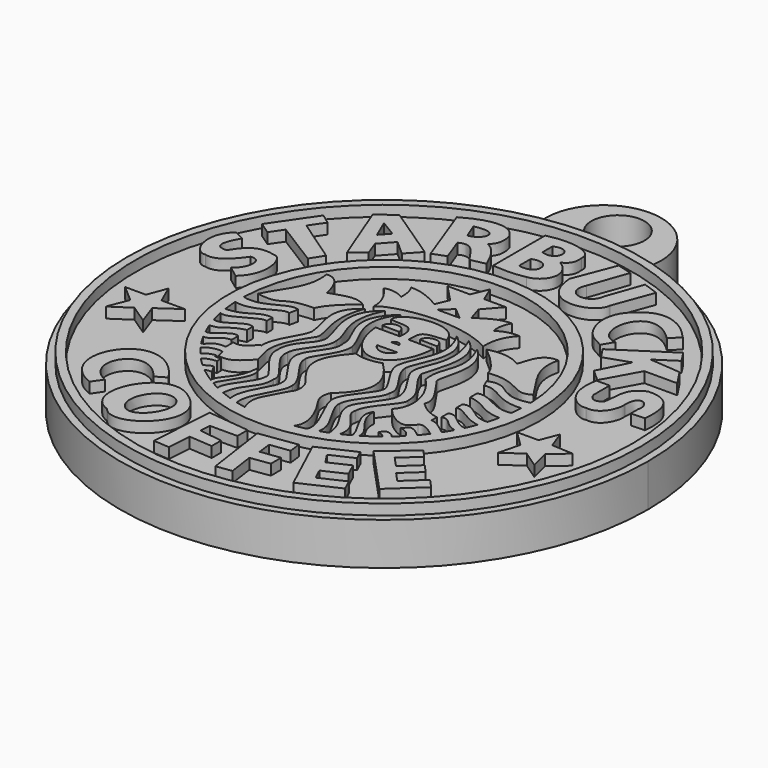
from build123d import *

# Parameters (mm, degrees)
F1_DEPTH = 6.35
F0_R     = 18.6234723368
F0_R_2   = 30.7555502211
F0_R_3   = 29.769220956
F2_DEPTH = 5.08
F3_DEPTH = 5.08
F4_D     = 6.35


with BuildPart() as f1:
    # F0 (on Top) → F1 (new body)
    with BuildSketch(Plane.XY):
        with BuildLine():
            add(Edge.make_bspline(
                [(-37.3034887016, 21.1265888065), (-35.8687117696, 21.2776176631), (-35.2645926178, 19.6729302406), (-34.9436551332, 18.2381533086)],
                knots=[0, 0, 0, 0, 3.7298624768, 3.7298624768, 3.7298624768, 3.7298624768], degree=3))
            add(Edge.make_bspline(
                [(-37.3034887016, 21.1265888065), (-36.8126444519, 17.9738514125), (-38.7949049473, 16.3502860814), (-39.8709885776, 14.0659688041)],
                knots=[0, 0, 0, 0, 7.5129495162, 7.5129495162, 7.5129495162, 7.5129495162], degree=3))
            add(Edge.make_bspline(
                [(-39.8709885776, 14.0659688041), (-36.4433825016, 13.4822865948), (-38.0642208973, 15.0488076413), (-33.9486729125, 15.0865653212)],
                knots=[0, 0, 0, 0, 6.0096123076, 6.0096123076, 6.0096123076, 6.0096123076], degree=3))
            add(Edge.make_bspline(
                [(-30.8169318073, 18.4591481001), (-32.0666968461, 17.530907802), (-33.3282358712, 16.4593721679), (-33.9486729125, 15.0865653212)],
                knots=[0, 0, 0, 0, 4.6024033885, 4.6024033885, 4.6024033885, 4.6024033885], degree=3))
            add(Edge.make_bspline(
                [(-34.9436551332, 18.2381533086), (-33.3956070244, 18.7478773296), (-32.0629240655, 19.3653249652), (-30.8169318073, 18.4591481001)],
                knots=[0, 0, 0, 0, 4.1326364596, 4.1326364596, 4.1326364596, 4.1326364596], degree=3))
        make_face()
    extrude(amount=F1_DEPTH)



with BuildPart() as f1b:
    # F0 (on Top) → F1, piece 2 (new body)
    with BuildSketch(Plane.XY):
        with Locations((-23.323516501, 12.2638461225)):
            Circle(F0_R)
        with BuildLine():
            ThreePointArc((-20.5316265155, -4.6995666709), (-23.5083377997, -4.9267869193), (-26.4794757553, -4.6356196819))
            ThreePointArc((-26.4794757553, -4.6356196819), (-27.0762181444, -4.5131993166), (-27.6682487288, -4.3697140845))
            ThreePointArc((-27.6682487288, -4.3697140845), (-28.1748264638, -4.2290861497), (-28.6768673036, -4.073034194))
            ThreePointArc((-28.6768673036, -4.073034194), (-29.2804679916, -3.86273914), (-29.8758340583, -3.6301514212))
            ThreePointArc((-29.8758340583, -3.6301514212), (-30.4056768992, -3.4012433245), (-30.9275370617, -3.1546782752))
            ThreePointArc((-30.9275370617, -3.1546782752), (-31.3412900052, -2.943630043), (-31.7491905199, -2.7214813887))
            ThreePointArc((-31.7491905199, -2.7214813887), (-32.0815979139, -2.5296670929), (-32.4096407461, -2.3304804975))
            ThreePointArc((-32.4096407461, -2.3304804975), (-33.2784322651, -1.7522758597), (-34.1105395793, -1.1224213333))
            ThreePointArc((-34.1105395793, -1.1224213333), (-34.5343783023, -0.7695187908), (-34.9466789077, -0.403202427))
            ThreePointArc((-34.9466789077, -0.403202427), (-35.4020262323, 0.0302192702), (-35.8412228525, 0.4799990857))
            ThreePointArc((-35.8412228525, 0.4799990857), (-36.1791670195, 0.8496324818), (-36.5062005914, 1.2289531252))
            ThreePointArc((-36.5062005914, 1.2289531252), (-36.8935004839, 1.7088682451), (-37.2633383656, 2.2023656314))
            ThreePointArc((-37.2633383656, 2.2023656314), (-37.5117320867, 2.5557792818), (-37.7511678916, 2.9153222476))
            ThreePointArc((-37.7511678916, 2.9153222476), (-38.1076469856, 3.4899354149), (-38.441253096, 4.0781229698))
            ThreePointArc((-38.441253096, 4.0781229698), (-38.688059763, 4.5513346225), (-38.9200586156, 5.0319793265))
            ThreePointArc((-38.9200586156, 5.0319793265), (-39.1883701818, 5.641275551), (-39.4328895696, 6.2605035015))
            ThreePointArc((-39.4328895696, 6.2605035015), (-39.6275252226, 6.8112024615), (-39.8033413414, 7.3681953469))
            ThreePointArc((-39.8033413414, 7.3681953469), (-40.0049668698, 8.1067754133), (-40.173508922, 8.8535999877))
            ThreePointArc((-40.173508922, 8.8535999877), (-40.2600967096, 9.3135454387), (-40.334132015, 9.775677494))
            ThreePointArc((-40.334132015, 9.775677494), (-40.4360379604, 10.6165354084), (-40.4964047471, 11.4613920264))
            ThreePointArc((-40.4964047471, 11.4613920264), (-40.5143834789, 12.1022421767), (-40.5084555729, 12.743317063))
            ThreePointArc((-40.5084555729, 12.743317063), (-23.3247020327, 29.4554726273), (-6.138643721, 12.7456871994))
            ThreePointArc((-6.138643721, 12.7456871994), (-6.1335784796, 12.504790326), (-6.1318899552, 12.2638461225))
            ThreePointArc((-6.1318899552, 12.2638461225), (-6.1381021555, 11.8017237781), (-6.1567342666, 11.3399354099))
            ThreePointArc((-6.1567342666, 11.3399354099), (-6.2057320104, 10.672156007), (-6.2806961413, 10.0067910778))
            ThreePointArc((-6.2806961413, 10.0067910778), (-6.394999893, 9.2676237104), (-6.5413466785, 8.5341277233))
            ThreePointArc((-6.5413466785, 8.5341277233), (-6.7054774656, 7.8601202107), (-6.8966661508, 7.1932829525))
            ThreePointArc((-6.8966661508, 7.1932829525), (-7.0638353358, 6.6804070661), (-7.2470130707, 6.1730283823))
            ThreePointArc((-7.2470130707, 6.1730283823), (-7.5036050003, 5.5346245183), (-7.7855363906, 4.9069991499))
            ThreePointArc((-7.7855363906, 4.9069991499), (-8.0117610702, 4.4470584884), (-8.2515967227, 3.9940663499))
            ThreePointArc((-8.2515967227, 3.9940663499), (-8.5617927331, 3.4522892402), (-8.891455006, 2.9221319172))
            ThreePointArc((-8.891455006, 2.9221319172), (-9.2140044154, 2.4417439038), (-9.5525375304, 1.9724826812))
            ThreePointArc((-9.5525375304, 1.9724826812), (-9.9356096896, 1.4788577359), (-10.3363666234, 0.9994792363))
            ThreePointArc((-10.3363666234, 0.9994792363), (-10.7036385779, 0.5894851337), (-11.0838477447, 0.1914589507))
            ThreePointArc((-11.0838477447, 0.1914589507), (-11.5686377385, -0.2810671322), (-12.0716556136, -0.7341402547))
            ThreePointArc((-12.0716556136, -0.7341402547), (-12.3762535826, -0.991698298), (-12.6867452193, -1.2421199662))
            ThreePointArc((-12.6867452193, -1.2421199662), (-13.5721120428, -1.8946189914), (-14.4973892188, -2.4891705347))
            ThreePointArc((-14.4973892188, -2.4891705347), (-14.7899052628, -2.6602787271), (-15.085737241, -2.8255878017))
            ThreePointArc((-15.085737241, -2.8255878017), (-15.6170587272, -3.1037344246), (-16.1577584837, -3.3631796767))
            ThreePointArc((-16.1577584837, -3.3631796767), (-16.6117176842, -3.563465081), (-17.0712677759, -3.7505664228))
            ThreePointArc((-17.0712677759, -3.7505664228), (-17.5593430337, -3.9326450879), (-18.052710843, -4.099852451))
            ThreePointArc((-18.052710843, -4.099852451), (-18.6457858767, -4.2791541948), (-19.2449367291, -4.4369685383))
            ThreePointArc((-19.2449367291, -4.4369685383), (-19.885773329, -4.5805578496), (-20.5316265155, -4.6995666709))
        make_face(mode=Mode.SUBTRACT)
        with BuildLine():
            add(Edge.make_bspline(
                [(-25.1541621983, 10.3296786547), (-24.256138131, 9.948018007), (-22.9764506221, 10.0153693929), (-21.9661723822, 10.3745795786)],
                knots=[0, 0, 0, 0, 3.1883060017, 3.1883060017, 3.1883060017, 3.1883060017], degree=3))
            add(Edge.make_bspline(
                [(-25.1541621983, 10.3296786547), (-28.2748024911, 6.8273791112), (-27.1747205406, 5.2782846615), (-25.1541621983, 2.7862638235)],
                knots=[0, 0, 0, 0, 7.5434148312, 7.5434148312, 7.5434148312, 7.5434148312], degree=3))
            add(Edge.make_bspline(
                [(-25.1541621983, 2.7862638235), (-24.7185155749, 2.0823951345), (-24.6232673526, 1.1775202584), (-25.1541621983, 0.5425201962)],
                knots=[0, 0, 0, 0, 2.2437436273, 2.2437436273, 2.2437436273, 2.2437436273], degree=3))
            add(Edge.make_bspline(
                [(-25.1541621983, 0.5425201962), (-26.2361075729, -1.6803713515), (-27.404530529, -2.5212091698), (-26.4794757553, -4.6356196819)],
                knots=[0, 0, 0, 0, 5.3450527239, 5.3450527239, 5.3450527239, 5.3450527239], degree=3))
            ThreePointArc((-26.4794757553, -4.6356196819), (-23.5083377997, -4.9267869193), (-20.5316265155, -4.6995666709))
            add(Edge.make_bspline(
                [(-21.9661723822, 0.7330201915), (-20.7424163818, -1.0196181247), (-19.5310563822, -3.4913323254), (-20.5316265155, -4.6995666709)],
                knots=[0, 0, 0, 0, 5.6188007494, 5.6188007494, 5.6188007494, 5.6188007494], degree=3))
            add(Edge.make_bspline(
                [(-21.9661723822, 2.6291091926), (-22.2737658769, 1.9871452823), (-22.3055165261, 1.3521452202), (-21.9661723822, 0.7330201915)],
                knots=[0, 0, 0, 0, 1.8960890011, 1.8960890011, 1.8960890011, 1.8960890011], degree=3))
            add(Edge.make_bspline(
                [(-21.9661723822, 10.3745795786), (-18.598575145, 7.1192374453), (-19.451700151, 4.8517226242), (-21.9661723822, 2.6291091926)],
                knots=[0, 0, 0, 0, 7.745470386, 7.745470386, 7.745470386, 7.745470386], degree=3))
        make_face()
        with BuildLine():
            add(Edge.make_bspline(
                [(-11.5920277312, 2.7170034591), (-11.1983073875, 3.228840651), (-9.9384002388, 2.2839105222), (-9.5525375304, 1.9724826812)],
                knots=[0, 0, 0, 0, 2.1711359857, 2.1711359857, 2.1711359857, 2.1711359857], degree=3))
            ThreePointArc((-9.5525375304, 1.9724826812), (-9.2140044154, 2.4417439038), (-8.891455006, 2.9221319172))
            add(Edge.make_bspline(
                [(-8.891455006, 2.9221319172), (-9.2555591837, 2.9907634016), (-10.2177355438, 4.1453759186), (-11.1799128354, 4.1774483398)],
                knots=[0, 0, 0, 0, 2.6101453135, 2.6101453135, 2.6101453135, 2.6101453135], degree=3))
            Line((-11.1799128354, 4.1774483398), (-11.1799128354, 4.9792625941))
            add(Edge.make_bspline(
                [(-11.1799128354, 4.9792625941), (-12.4948881567, 5.2358433604), (-13.0721945316, 5.7490044273), (-13.8098634779, 6.4225285314)],
                knots=[0, 0, 0, 0, 2.9999428241, 2.9999428241, 2.9999428241, 2.9999428241], degree=3))
            add(Edge.make_bspline(
                [(-13.8098634779, 6.4225285314), (-13.245656155, 7.5597707182), (-14.8599110544, 9.2527708039), (-15.7654695213, 10.7095381245)],
                knots=[0, 0, 0, 0, 4.7119896273, 4.7119896273, 4.7119896273, 4.7119896273], degree=3))
            add(Edge.make_bspline(
                [(-15.7654695213, 10.7095381245), (-16.159189865, 11.7332125083), (-13.6787490919, 15.3160719201), (-16.789143905, 18.0327463895)],
                knots=[0, 0, 0, 0, 7.3944092757, 7.3944092757, 7.3944092757, 7.3944092757], degree=3))
            add(Edge.make_bspline(
                [(-16.789143905, 18.0327463895), (-14.8599110544, 13.8593045995), (-17.3403527588, 13.1899798289), (-16.789143905, 10.3158168495)],
                knots=[0, 0, 0, 0, 7.71692954, 7.71692954, 7.71692954, 7.71692954], degree=3))
            add(Edge.make_bspline(
                [(-16.789143905, 10.3158168495), (-14.3480747938, 7.7960030176), (-14.1905862838, 5.0005847588), (-15.4898650944, 3.7013057154)],
                knots=[0, 0, 0, 0, 6.740911138, 6.740911138, 6.740911138, 6.740911138], degree=3))
            add(Edge.make_bspline(
                [(-15.4898650944, 3.7013057154), (-14.8599110544, 2.7170034591), (-13.0487950519, 1.4177246485), (-12.2613534331, 2.04767799)],
                knots=[0, 0, 0, 0, 3.6273643601, 3.6273643601, 3.6273643601, 3.6273643601], degree=3))
            Line((-12.2613534331, 2.04767799), (-11.5920277312, 2.7170034591))
        make_face()
        with BuildLine():
            ThreePointArc((-37.7511678916, 2.9153222476), (-37.5117320867, 2.5557792818), (-37.2633383656, 2.2023656314))
            add(Edge.make_bspline(
                [(-35.1136736572, 2.8264259454), (-35.7692502439, 3.1008527149), (-36.9269598619, 2.6530623946), (-37.2633383656, 2.2023656314)],
                knots=[0, 0, 0, 0, 2.2384167695, 2.2384167695, 2.2384167695, 2.2384167695], degree=3))
            Line((-35.1136736572, 2.8264259454), (-34.8849855363, 1.9421626348))
            add(Edge.make_bspline(
                [(-34.8849855363, 1.9421626348), (-33.1683903933, 1.578410971), (-32.4025005102, 2.9314819258), (-31.5461270511, 3.6497057881)],
                knots=[0, 0, 0, 0, 3.7501572773, 3.7501572773, 3.7501572773, 3.7501572773], degree=3))
            add(Edge.make_bspline(
                [(-31.5461270511, 3.6497057881), (-32.0893339813, 5.675278604), (-32.8234881163, 6.5929680131), (-30.1621854305, 10.6308031827)],
                knots=[0, 0, 0, 0, 7.1169526654, 7.1169526654, 7.1169526654, 7.1169526654], degree=3))
            add(Edge.make_bspline(
                [(-30.1621854305, 10.6308031827), (-29.5198019594, 11.4108398557), (-31.7222587764, 14.1180250794), (-30.141601339, 17.9168451577)],
                knots=[0, 0, 0, 0, 7.2860710514, 7.2860710514, 7.2860710514, 7.2860710514], degree=3))
            add(Edge.make_bspline(
                [(-31.1447884887, 11.1646270379), (-31.183373183, 13.2481688634), (-33.1897474825, 15.7947186381), (-30.141601339, 17.9168451577)],
                knots=[0, 0, 0, 0, 6.826333862, 6.826333862, 6.826333862, 6.826333862], degree=3))
            add(Edge.make_bspline(
                [(-33.0595215658, 6.1291290476), (-33.2283303142, 7.8078093939), (-31.3762910664, 9.8913516849), (-31.1447884887, 11.1646270379)],
                knots=[0, 0, 0, 0, 5.3872481628, 5.3872481628, 5.3872481628, 5.3872481628], degree=3))
            add(Edge.make_bspline(
                [(-35.5113420169, 4.9364422448), (-34.1983001212, 4.5602791943), (-33.7350321809, 5.8482989697), (-33.0595215658, 6.1291290476)],
                knots=[0, 0, 0, 0, 2.7265225716, 2.7265225716, 2.7265225716, 2.7265225716], degree=3))
            Line((-35.5113420169, 4.9364422448), (-35.5113420169, 3.7996245127))
            add(Edge.make_bspline(
                [(-35.5113420169, 3.7996245127), (-37.2722457627, 3.9979689799), (-37.2112627606, 2.801016676), (-37.7511678916, 2.9153222476)],
                knots=[0, 0, 0, 0, 2.4080719353, 2.4080719353, 2.4080719353, 2.4080719353], degree=3))
        make_face()
        with BuildLine():
            add(Edge.make_bspline(
                [(-19.0454814583, 1.2633221922), (-18.9428050071, -0.5164264585), (-17.2315072268, -1.3036229648), (-17.0712677759, -3.7505664228)],
                knots=[0, 0, 0, 0, 5.3885618404, 5.3885618404, 5.3885618404, 5.3885618404], degree=3))
            ThreePointArc((-17.0712677759, -3.7505664228), (-16.6117176842, -3.563465081), (-16.1577584837, -3.3631796767))
            add(Edge.make_bspline(
                [(-16.1577584837, -3.3631796767), (-15.4627067968, -1.1172490194), (-18.4270944446, 0), (-17.9378278553, 1.2139687315)],
                knots=[0, 0, 0, 0, 4.9111031875, 4.9111031875, 4.9111031875, 4.9111031875], degree=3))
            add(Edge.make_bspline(
                [(-17.9378278553, 1.2139687315), (-17.9666075855, 2.8544552624), (-15.2324633673, 4.9266489223), (-15.3763657436, 5.9051848948)],
                knots=[0, 0, 0, 0, 5.344959985, 5.344959985, 5.344959985, 5.344959985], degree=3))
            add(Edge.make_bspline(
                [(-15.3763657436, 5.9051848948), (-15.3693296015, 8.0646779388), (-16.9094968587, 8.5096154362), (-17.7993699908, 10.8712045476)],
                knots=[0, 0, 0, 0, 5.5256041094, 5.5256041094, 5.5256041094, 5.5256041094], degree=3))
            add(Edge.make_bspline(
                [(-17.7993699908, 10.8712045476), (-17.3886585981, 12.7878570929), (-15.4377808794, 16.7005695403), (-18.4838883579, 18.8910309225)],
                knots=[0, 0, 0, 0, 8.0489863013, 8.0489863013, 8.0489863013, 8.0489863013], degree=3))
            add(Edge.make_bspline(
                [(-18.4838883579, 18.8910309225), (-16.4303332567, 14.5443370566), (-18.930003047, 12.477661483), (-18.7919232994, 10.9396567568)],
                knots=[0, 0, 0, 0, 7.9573385405, 7.9573385405, 7.9573385405, 7.9573385405], degree=3))
            add(Edge.make_bspline(
                [(-18.7919232994, 10.9396567568), (-18.8401266932, 9.6486760303), (-16.3074079901, 7.5266682543), (-16.6496671736, 5.8838231489)],
                knots=[0, 0, 0, 0, 5.4909666526, 5.4909666526, 5.4909666526, 5.4909666526], degree=3))
            add(Edge.make_bspline(
                [(-16.6496671736, 5.8838231489), (-16.7181193829, 4.6516899019), (-19.250838086, 2.4612299167), (-19.0454814583, 1.2633221922)],
                knots=[0, 0, 0, 0, 5.2047050999, 5.2047050999, 5.2047050999, 5.2047050999], degree=3))
        make_face()
        with BuildLine():
            ThreePointArc((-30.9275370617, -3.1546782752), (-30.4056768992, -3.4012433245), (-29.8758340583, -3.6301514212))
            add(Edge.make_bspline(
                [(-27.9058404267, 1.4696465805), (-27.6762954891, -0.7835272118), (-29.8235695809, -1.2996989535), (-29.8758340583, -3.6301514212)],
                knots=[0, 0, 0, 0, 5.4670663584, 5.4670663584, 5.4670663584, 5.4670663584], degree=3))
            add(Edge.make_bspline(
                [(-30.2663836628, 6.4466488548), (-30.755110085, 4.8970277421), (-27.4103153497, 2.5845777709), (-27.9058404267, 1.4696465805)],
                knots=[0, 0, 0, 0, 5.5084222793, 5.5084222793, 5.5084222793, 5.5084222793], degree=3))
            add(Edge.make_bspline(
                [(-28.2149165869, 11.3540776074), (-27.8152227402, 9.496984072), (-30.3753241897, 7.8810332343), (-30.2663836628, 6.4466488548)],
                knots=[0, 0, 0, 0, 5.3189636327, 5.3189636327, 5.3189636327, 5.3189636327], degree=3))
            add(Edge.make_bspline(
                [(-28.4327305853, 18.7597032636), (-30.4172430187, 14.6938692778), (-28.1668771058, 12.9488036036), (-28.2149165869, 11.3540776074)],
                knots=[0, 0, 0, 0, 7.4088281326, 7.4088281326, 7.4088281326, 7.4088281326], degree=3))
            add(Edge.make_bspline(
                [(-29.2691271752, 11.3491620868), (-29.4733904302, 13.0239734426), (-31.6999182105, 16.2669606507), (-28.4327305853, 18.7597032636)],
                knots=[0, 0, 0, 0, 7.4575920905, 7.4575920905, 7.4575920905, 7.4575920905], degree=3))
            add(Edge.make_bspline(
                [(-31.3623659313, 6.3486085273), (-31.4714536071, 8.880619891), (-28.8093015552, 9.5582595095), (-29.2691271752, 11.3491620868)],
                knots=[0, 0, 0, 0, 5.4209947788, 5.4209947788, 5.4209947788, 5.4209947788], degree=3))
            add(Edge.make_bspline(
                [(-28.7954192609, 1.4543000143), (-28.5216122866, 2.1045927424), (-31.5677188337, 4.4319564477), (-31.3623659313, 6.3486085273)],
                knots=[0, 0, 0, 0, 5.5266147893, 5.5266147893, 5.5266147893, 5.5266147893], degree=3))
            add(Edge.make_bspline(
                [(-30.9275370617, -3.1546782752), (-31.0885570943, -1.7971637426), (-28.7611931562, 0), (-28.7954192609, 1.4543000143)],
                knots=[0, 0, 0, 0, 5.0782484372, 5.0782484372, 5.0782484372, 5.0782484372], degree=3))
        make_face()
        with BuildLine():
            ThreePointArc((-28.6768673036, -4.073034194), (-28.1748264638, -4.2290861497), (-27.6682487288, -4.3697140845))
            add(Edge.make_bspline(
                [(-27.6682487288, -4.3697140845), (-28.0305817723, -2.2636251524), (-25.5194604397, 0), (-25.7530529052, 1.561455545)],
                knots=[0, 0, 0, 0, 6.2327159583, 6.2327159583, 6.2327159583, 6.2327159583], degree=3))
            add(Edge.make_bspline(
                [(-25.7530529052, 1.561455545), (-25.7822517306, 3.2258036081), (-28.3225737512, 5.1237442531), (-28.1473789364, 6.5253004432)],
                knots=[0, 0, 0, 0, 5.5111299492, 5.5111299492, 5.5111299492, 5.5111299492], degree=3))
            add(Edge.make_bspline(
                [(-28.1473789364, 6.5253004432), (-28.3412262797, 7.3351999745), (-25.9595457464, 9.5450067893), (-26.3032950461, 11.2637449056)],
                knots=[0, 0, 0, 0, 5.0846338431, 5.0846338431, 5.0846338431, 5.0846338431], degree=3))
            add(Edge.make_bspline(
                [(-26.3032950461, 11.2637449056), (-26.8041826785, 13.3823882788), (-29.3643958867, 15.4883693904), (-26.8041826785, 19.0602783114)],
                knots=[0, 0, 0, 0, 7.8126065796, 7.8126065796, 7.8126065796, 7.8126065796], degree=3))
            add(Edge.make_bspline(
                [(-26.8041826785, 19.0602783114), (-30.8303236961, 15.4677229002), (-26.9900038838, 12.9694510251), (-27.3616481572, 11.2144667655)],
                knots=[0, 0, 0, 0, 7.8655913047, 7.8655913047, 7.8655913047, 7.8655913047], degree=3))
            add(Edge.make_bspline(
                [(-27.3616481572, 11.2144667655), (-26.8892925233, 9.4300266355), (-29.4674020261, 8.0550359562), (-29.2955264449, 6.2871901318)],
                knots=[0, 0, 0, 0, 5.2931975456, 5.2931975456, 5.2931975456, 5.2931975456], degree=3))
            add(Edge.make_bspline(
                [(-29.2955264449, 6.2871901318), (-29.1757863015, 4.5045078732), (-26.6828406602, 2.4702642113), (-26.9221644849, 1.6126909759)],
                knots=[0, 0, 0, 0, 5.2424983884, 5.2424983884, 5.2424983884, 5.2424983884], degree=3))
            add(Edge.make_bspline(
                [(-26.9221644849, 1.6126909759), (-26.6030672938, 0.33630291), (-29.0561262518, -1.8973762635), (-28.6768673036, -4.073034194)],
                knots=[0, 0, 0, 0, 5.9503321495, 5.9503321495, 5.9503321495, 5.9503321495], degree=3))
        make_face()
        with BuildLine():
            add(Edge.make_bspline(
                [(-21.0185293108, 1.3900708873), (-20.917724818, 0), (-18.5001660138, -3.1988520641), (-19.2449367291, -4.4369685383)],
                knots=[0, 0, 0, 0, 6.0909785021, 6.0909785021, 6.0909785021, 6.0909785021], degree=3))
            ThreePointArc((-19.2449367291, -4.4369685383), (-18.6457858767, -4.2791541948), (-18.052710843, -4.099852451))
            add(Edge.make_bspline(
                [(-18.052710843, -4.099852451), (-17.6375582814, -2.1530971862), (-20.1414600015, 0), (-19.9975576252, 1.4156807447)],
                knots=[0, 0, 0, 0, 5.8483788728, 5.8483788728, 5.8483788728, 5.8483788728], degree=3))
            add(Edge.make_bspline(
                [(-19.9975576252, 1.4156807447), (-19.9975576252, 2.9698258732), (-17.5512172282, 4.7542145476), (-17.6663398743, 6.0781161301)],
                knots=[0, 0, 0, 0, 5.2127612573, 5.2127612573, 5.2127612573, 5.2127612573], degree=3))
            add(Edge.make_bspline(
                [(-17.6663398743, 6.0781161301), (-17.1613674611, 7.3881517164), (-19.6940470487, 9.2588821426), (-19.6940470487, 10.9569299966)],
                knots=[0, 0, 0, 0, 5.2834099907, 5.2834099907, 5.2834099907, 5.2834099907], degree=3))
            add(Edge.make_bspline(
                [(-19.6940470487, 10.9569299966), (-19.4866359234, 12.8164812922), (-16.437260434, 16.228877008), (-19.9706628919, 18.9636349678)],
                knots=[0, 0, 0, 0, 8.0114818118, 8.0114818118, 8.0114818118, 8.0114818118], degree=3))
            add(Edge.make_bspline(
                [(-19.9706628919, 18.9636349678), (-17.8651418537, 15.4302315786), (-20.1642736793, 13.5183213279), (-20.5998998135, 11.0981827602)],
                knots=[0, 0, 0, 0, 7.8905815713, 7.8905815713, 7.8905815713, 7.8905815713], degree=3))
            add(Edge.make_bspline(
                [(-20.5998998135, 11.0981827602), (-20.9609698504, 9.563723579), (-18.2843860239, 7.1192374453), (-18.598575145, 6.1964089982)],
                knots=[0, 0, 0, 0, 5.2945902998, 5.2945902998, 5.2945902998, 5.2945902998], degree=3))
            add(Edge.make_bspline(
                [(-18.598575145, 6.1964089982), (-18.7736526132, 5.1315315068), (-21.5077977628, 2.8003137559), (-21.0185293108, 1.3900708873)],
                knots=[0, 0, 0, 0, 5.3811768417, 5.3811768417, 5.3811768417, 5.3811768417], degree=3))
        make_face()
        with BuildLine():
            ThreePointArc((-40.5084555729, 12.743317063), (-40.5143834789, 12.1022421767), (-40.4964047471, 11.4613920264))
            add(Edge.make_bspline(
                [(-35.1534485817, 12.8513416275), (-36.2611077726, 13.2579505444), (-37.9218748563, 10.8747574392), (-40.4964047471, 11.4613920264)],
                knots=[0, 0, 0, 0, 5.5207916533, 5.5207916533, 5.5207916533, 5.5207916533], degree=3))
            Line((-35.1534485817, 12.8513416275), (-34.9291153252, 13.9169376343))
            add(Edge.make_bspline(
                [(-34.9291153252, 13.9169376343), (-36.471426487, 14.5058203489), (-37.937392151, 12.0239456985), (-40.5084555729, 12.743317063)],
                knots=[0, 0, 0, 0, 5.7014404185, 5.7014404185, 5.7014404185, 5.7014404185], degree=3))
        make_face()
        with BuildLine():
            add(Edge.make_bspline(
                [(-11.2570207566, 10.0684184581), (-9.1691110283, 9.8439119756), (-9.0119568631, 8.6315777153), (-6.5413466785, 8.5341277233)],
                knots=[0, 0, 0, 0, 4.9589948649, 4.9589948649, 4.9589948649, 4.9589948649], degree=3))
            ThreePointArc((-6.5413466785, 8.5341277233), (-6.394999893, 9.2676237104), (-6.2806961413, 10.0067910778))
            add(Edge.make_bspline(
                [(-11.2570207566, 11.1011480913), (-9.8201790825, 11.6399638355), (-8.3833392709, 9.5520541072), (-6.2806961413, 10.0067910778)],
                knots=[0, 0, 0, 0, 5.0952354166, 5.0952354166, 5.0952354166, 5.0952354166], degree=3))
            Line((-11.2570207566, 11.1011480913), (-11.2570207566, 10.0684184581))
        make_face()
        with BuildLine():
            add(Edge.make_bspline(
                [(-11.7509346455, 12.7624953166), (-9.932433255, 13.1217055023), (-9.3038147315, 11.1235985532), (-6.1567342666, 11.3399354099)],
                knots=[0, 0, 0, 0, 5.7722399957, 5.7722399957, 5.7722399957, 5.7722399957], degree=3))
            ThreePointArc((-6.1567342666, 11.3399354099), (-6.1381021555, 11.8017237781), (-6.1318899552, 12.2638461225))
            ThreePointArc((-6.1318899552, 12.2638461225), (-6.1335784796, 12.504790326), (-6.138643721, 12.7456871994))
            add(Edge.make_bspline(
                [(-12.1101448312, 13.6156203225), (-9.4834202901, 14.6258985624), (-9.932433255, 11.7746675387), (-6.138643721, 12.7456871994)],
                knots=[0, 0, 0, 0, 6.0345347085, 6.0345347085, 6.0345347085, 6.0345347085], degree=3))
            Line((-12.1101448312, 13.6156203225), (-11.7509346455, 12.7624953166))
        make_face()
        with BuildLine():
            ThreePointArc((-40.334132015, 9.775677494), (-40.2600967096, 9.3135454387), (-40.173508922, 8.8535999877))
            add(Edge.make_bspline(
                [(-35.7946865261, 10.2548254654), (-36.5283489227, 10.7307136059), (-39.1763295122, 8.2058338933), (-40.173508922, 8.8535999877)],
                knots=[0, 0, 0, 0, 4.5975557, 4.5975557, 4.5975557, 4.5975557], degree=3))
            Line((-35.7946865261, 10.2548254654), (-35.7946865261, 11.127287522))
            add(Edge.make_bspline(
                [(-35.7946865261, 11.127287522), (-37.5495254993, 11.4346323535), (-37.9168383976, 9.8001597316), (-40.334132015, 9.775677494)],
                knots=[0, 0, 0, 0, 4.7363926162, 4.7363926162, 4.7363926162, 4.7363926162], degree=3))
        make_face()
        with BuildLine():
            add(Edge.make_bspline(
                [(-10.9427124262, 7.5539466925), (-10.2082267404, 7.9564619809), (-9.051611647, 6.414307747), (-7.2470130707, 6.1730283823)],
                knots=[0, 0, 0, 0, 3.9452666711, 3.9452666711, 3.9452666711, 3.9452666711], degree=3))
            ThreePointArc((-7.2470130707, 6.1730283823), (-7.0638353358, 6.6804070661), (-6.8966661508, 7.1932829525))
            add(Edge.make_bspline(
                [(-10.9427124262, 8.541774936), (-9.4598289579, 9.0677198023), (-8.8701825589, 6.9585973397), (-6.8966661508, 7.1932829525)],
                knots=[0, 0, 0, 0, 4.2648471359, 4.2648471359, 4.2648471359, 4.2648471359], degree=3))
            Line((-10.9427124262, 8.541774936), (-10.9427124262, 7.5539466925))
        make_face()
        with BuildLine():
            ThreePointArc((-39.8033413414, 7.3681953469), (-39.6275252226, 6.8112024615), (-39.4328895696, 6.2605035015))
            add(Edge.make_bspline(
                [(-36.0845923424, 7.6848659664), (-38.0627140403, 7.2857607156), (-37.9144308218, 6.237241817), (-39.4328895696, 6.2605035015)],
                knots=[0, 0, 0, 0, 3.6386677168, 3.6386677168, 3.6386677168, 3.6386677168], degree=3))
            Line((-36.0845923424, 7.6848659664), (-36.0845923424, 8.573836647))
            add(Edge.make_bspline(
                [(-36.0845923424, 8.573836647), (-37.2768603265, 9.0758437291), (-38.3914488678, 7.085816014), (-39.8033413414, 7.3681953469)],
                knots=[0, 0, 0, 0, 3.9093049334, 3.9093049334, 3.9093049334, 3.9093049334], degree=3))
        make_face()
        with BuildLine():
            ThreePointArc((-32.4096407461, -2.3304804975), (-32.0815979139, -2.5296670929), (-31.7491905199, -2.7214813887))
            add(Edge.make_bspline(
                [(-30.482897535, 2.2050866392), (-28.7271812558, 1.0157307843), (-32.2197340429, -2.1936418489), (-31.7491905199, -2.7214813887)],
                knots=[0, 0, 0, 0, 5.0867052653, 5.0867052653, 5.0867052653, 5.0867052653], degree=3))
            add(Edge.make_bspline(
                [(-30.482897535, 2.2050866392), (-30.615048483, -0.6267128629), (-32.4462801218, -1.0986793786), (-32.4096407461, -2.3304804975)],
                knots=[0, 0, 0, 0, 4.9278503075, 4.9278503075, 4.9278503075, 4.9278503075], degree=3))
        make_face()
        with BuildLine():
            add(Edge.make_bspline(
                [(-10.8432313427, 5.2576926537), (-9.8000103608, 5.5525163189), (-9.8226889968, 4.3732221238), (-8.2515967227, 3.9940663499)],
                knots=[0, 0, 0, 0, 2.8832831008, 2.8832831008, 2.8832831008, 2.8832831008], degree=3))
            ThreePointArc((-8.2515967227, 3.9940663499), (-8.0117610702, 4.4470584884), (-7.7855363906, 4.9069991499))
            add(Edge.make_bspline(
                [(-10.8432313427, 6.2782354653), (-9.7319735214, 6.6637741402), (-9.2103630304, 5.0762626342), (-7.7855363906, 4.9069991499)],
                knots=[0, 0, 0, 0, 3.351087503, 3.351087503, 3.351087503, 3.351087503], degree=3))
            Line((-10.8432313427, 6.2782354653), (-10.8432313427, 5.2576926537))
        make_face()
        with BuildLine():
            ThreePointArc((-38.9200586156, 5.0319793265), (-38.688059763, 4.5513346225), (-38.441253096, 4.0781229698))
            add(Edge.make_bspline(
                [(-35.9678204636, 5.2481344946), (-37.2789699117, 5.2176425278), (-37.5229056458, 3.9979689799), (-38.441253096, 4.0781229698)],
                knots=[0, 0, 0, 0, 2.7362010078, 2.7362010078, 2.7362010078, 2.7362010078], degree=3))
            Line((-35.9678204636, 5.2481344946), (-35.9678204636, 6.2187905423))
            add(Edge.make_bspline(
                [(-35.9678204636, 6.2187905423), (-36.8368375579, 6.8438732997), (-38.3270053415, 4.629806351), (-38.9200586156, 5.0319793265)],
                knots=[0, 0, 0, 0, 3.1818596714, 3.1818596714, 3.1818596714, 3.1818596714], degree=3))
        make_face()
        with BuildLine():
            add(Edge.make_bspline(
                [(-16.4414569736, 2.134141745), (-17.6002308726, 0.7767199422), (-15.2164660394, -1.3421825133), (-15.085737241, -2.8255878017)],
                knots=[0, 0, 0, 0, 5.1416819398, 5.1416819398, 5.1416819398, 5.1416819398], degree=3))
            ThreePointArc((-15.085737241, -2.8255878017), (-14.7899052628, -2.6602787271), (-14.4973892188, -2.4891705347))
            add(Edge.make_bspline(
                [(-16.4414569736, 2.134141745), (-16.6590125925, 0), (-14.2894461751, -1.1435353663), (-14.4973892188, -2.4891705347)],
                knots=[0, 0, 0, 0, 5.0154178162, 5.0154178162, 5.0154178162, 5.0154178162], degree=3))
        make_face()
        with BuildLine():
            ThreePointArc((-36.5062005914, 1.2289531252), (-36.1791670195, 0.8496324818), (-35.8412228525, 0.4799990857))
            add(Edge.make_bspline(
                [(-34.3487411737, 1.0153454496), (-35.5167724192, 0.9342323174), (-35.5223989356, 0.6548584507), (-35.8412228525, 0.4799990857)],
                knots=[0, 0, 0, 0, 1.585590518, 1.585590518, 1.585590518, 1.585590518], degree=3))
            Line((-34.3487411737, 1.0153454496), (-34.3487411737, 1.6318048583))
            Line((-34.3487411737, 1.6318048583), (-35.0949838758, 1.6318048583))
            Line((-35.0949838758, 1.6318048583), (-35.0949838758, 1.8913667882))
            add(Edge.make_bspline(
                [(-35.0949838758, 1.8913667882), (-35.5978831649, 1.8751441967), (-36.1332297325, 1.6480274498), (-36.5062005914, 1.2289531252)],
                knots=[0, 0, 0, 0, 1.5589498002, 1.5589498002, 1.5589498002, 1.5589498002], degree=3))
        make_face()
        with BuildLine():
            add(Edge.make_bspline(
                [(-12.4519607052, 1.1574601522), (-11.5746026859, 1.0415826691), (-11.2766325474, 0.5615188857), (-11.0838477447, 0.1914589507)],
                knots=[0, 0, 0, 0, 1.6747809988, 1.6747809988, 1.6747809988, 1.6747809988], degree=3))
            ThreePointArc((-11.0838477447, 0.1914589507), (-10.7036385779, 0.5894851337), (-10.3363666234, 0.9994792363))
            add(Edge.make_bspline(
                [(-11.8229119107, 1.8361710245), (-11.2600782886, 1.7368475674), (-10.6972446665, 1.3561072992), (-10.3363666234, 0.9994792363)],
                knots=[0, 0, 0, 0, 1.7058341184, 1.7058341184, 1.7058341184, 1.7058341184], degree=3))
            Line((-11.8229119107, 1.8361710245), (-12.4519607052, 1.1574601522))
        make_face()
        with BuildLine():
            ThreePointArc((-34.9466789077, -0.403202427), (-34.5343783023, -0.7695187908), (-34.1105395793, -1.1224213333))
            add(Edge.make_bspline(
                [(-33.3610139787, -0.9467520867), (-33.5330814123, -0.9696943453), (-34.0836942196, -0.9811654454), (-34.1105395793, -1.1224213333)],
                knots=[0, 0, 0, 0, 0.7698365476, 0.7698365476, 0.7698365476, 0.7698365476], degree=3))
            Line((-33.3610139787, -0.9467520867), (-33.8657461107, -0.052004496))
            add(Edge.make_bspline(
                [(-33.8657461107, -0.052004496), (-34.4278290868, 0), (-34.4278290868, -0.3273114562), (-34.9466789077, -0.403202427)],
                knots=[0, 0, 0, 0, 1.1365543095, 1.1365543095, 1.1365543095, 1.1365543095], degree=3))
        make_face()
        with BuildLine():
            add(Edge.make_bspline(
                [(-13.5941812769, -0.7627950399), (-13.2134407759, -0.9283344261), (-12.9320248961, -0.9448883357), (-12.6867452193, -1.2421199662)],
                knots=[0, 0, 0, 0, 1.0262517155, 1.0262517155, 1.0262517155, 1.0262517155], degree=3))
            ThreePointArc((-12.6867452193, -1.2421199662), (-12.3762535826, -0.991698298), (-12.0716556136, -0.7341402547))
            add(Edge.make_bspline(
                [(-13.0644561723, -0.2165155456), (-12.5512843952, -0.2165155456), (-12.137436308, -0.4151626199), (-12.0716556136, -0.7341402547)],
                knots=[0, 0, 0, 0, 1.1196375702, 1.1196375702, 1.1196375702, 1.1196375702], degree=3))
            Line((-13.0644561723, -0.2165155456), (-13.5941812769, -0.7627950399))
        make_face()
    extrude(amount=F1_DEPTH)


with BuildPart() as f1c:
    # F0 (on Top) → F1, piece 3 (new body)
    with BuildSketch(Plane.XY):
        with BuildLine():
            Line((-22.6796176285, 26.4355707914), (-23.4705228359, 28.3249542117))
            Line((-23.4705228359, 28.3249542117), (-24.3053659797, 26.3476930559))
            Line((-24.3053659797, 26.3476930559), (-26.9856527448, 26.3476930559))
            Line((-26.9856527448, 26.3476930559), (-25.0095480739, 24.2618030685))
            Line((-25.0095480739, 24.2618030685), (-25.6674792618, 22.7227136493))
            add(Edge.make_bspline(
                [(-29.4629596174, 24.0147784352), (-28.1827673316, 24.0409038961), (-26.9025750458, 23.4399978071), (-25.6674792618, 22.7227136493)],
                knots=[0, 0, 0, 0, 4.009376827, 4.009376827, 4.009376827, 4.009376827], degree=3))
            add(Edge.make_bspline(
                [(-29.4629596174, 24.0147784352), (-29.1494429111, 23.466123268), (-28.9665590972, 22.6300805807), (-29.0188118815, 21.9246670604)],
                knots=[0, 0, 0, 0, 2.1367809365, 2.1367809365, 2.1367809365, 2.1367809365], degree=3))
            add(Edge.make_bspline(
                [(-31.3701853156, 22.2643110901), (-30.8737829328, 22.525575012), (-29.8026017845, 22.4471949041), (-29.0188118815, 21.9246670604)],
                knots=[0, 0, 0, 0, 2.3757767347, 2.3757767347, 2.3757767347, 2.3757767347], degree=3))
            add(Edge.make_bspline(
                [(-31.3701853156, 22.2643110901), (-30.5602662265, 21.4282665402), (-29.7242235392, 20.1742015779), (-29.828729108, 18.8156310469)],
                knots=[0, 0, 0, 0, 3.777496695, 3.777496695, 3.777496695, 3.777496695], degree=3))
            add(Edge.make_bspline(
                [(-29.828729108, 18.8156310469), (-28.6269150674, 20.1219487935), (-21.5727966279, 21.5850248933), (-16.765544191, 18.8940092921)],
                knots=[0, 0, 0, 0, 13.063420047, 13.063420047, 13.063420047, 13.063420047], degree=3))
            add(Edge.make_bspline(
                [(-16.765544191, 18.8940092921), (-16.8321467936, 20.3368868679), (-16.444189474, 21.5377062559), (-15.4096381739, 22.6461533457)],
                knots=[0, 0, 0, 0, 3.9896197972, 3.9896197972, 3.9896197972, 3.9896197972], degree=3))
            add(Edge.make_bspline(
                [(-15.4096381739, 22.6461533457), (-16.3887664676, 22.7200500667), (-17.1462055296, 22.4798861891), (-17.959067598, 21.9626110047)],
                knots=[0, 0, 0, 0, 2.6394735309, 2.6394735309, 2.6394735309, 2.6394735309], degree=3))
            add(Edge.make_bspline(
                [(-17.959067598, 21.9626110047), (-18.1622840464, 22.8493697941), (-17.8482234478, 23.8100234419), (-17.5341628492, 24.2164544761)],
                knots=[0, 0, 0, 0, 2.2935462583, 2.2935462583, 2.2935462583, 2.2935462583], degree=3))
            add(Edge.make_bspline(
                [(-21.2296266109, 22.7446835488), (-20.1205424964, 23.4405416995), (-19.0490409732, 24.2164544761), (-17.5341628492, 24.2164544761)],
                knots=[0, 0, 0, 0, 3.9777584236, 3.9777584236, 3.9777584236, 3.9777584236], degree=3))
            Line((-21.2296266109, 22.7446835488), (-21.778864786, 24.4802795351))
            Line((-21.778864786, 24.4802795351), (-20.0652386993, 26.4355707914))
            Line((-20.0652386993, 26.4355707914), (-22.6796176285, 26.4355707914))
        make_face()
        Polygon((-24.7227884829, 22.01968804), (-23.4705228359, 23.2060439885), (-22.0864396542, 22.01968804), align=None, mode=Mode.SUBTRACT)
    extrude(amount=F1_DEPTH)


with BuildPart() as f1d:
    # F0 (on Top) → F1, piece 4 (new body)
    with BuildSketch(Plane.XY):
        with BuildLine():
            add(Edge.make_bspline(
                [(-26.9022230059, 17.7935324609), (-27.2212196141, 19.6809303015), (-20.9488011897, 21.0450235754), (-20.2576424927, 17.7487246692)],
                knots=[0, 0, 0, 0, 6.6447315924, 6.6447315924, 6.6447315924, 6.6447315924], degree=3))
            add(Edge.make_bspline(
                [(-26.9022230059, 17.7935324609), (-25.5996547639, 17.4479521811), (-23.818589747, 18.3517765254), (-24.1110026836, 15.6137226149)],
                knots=[0, 0, 0, 0, 3.5415366512, 3.5415366512, 3.5415366512, 3.5415366512], degree=3))
            Line((-24.1110026836, 15.6137226149), (-27.0386859775, 15.6074939296))
            add(Edge.make_bspline(
                [(-27.0386859775, 15.6074939296), (-26.3863280416, 9.2225940898), (-20.5423012379, 8.8858669624), (-20.0764741751, 15.5718578026)],
                knots=[0, 0, 0, 0, 6.9623030036, 6.9623030036, 6.9623030036, 6.9623030036], degree=3))
            Line((-20.0764741751, 15.5718578026), (-23.0801980942, 15.6040266156))
            add(Edge.make_bspline(
                [(-20.2576424927, 17.7487246692), (-23.0246353894, 17.5153631717), (-23.0246353894, 17.5153631717), (-23.0801980942, 15.6040266156)],
                knots=[0, 0, 0, 0, 3.5449329846, 3.5449329846, 3.5449329846, 3.5449329846], degree=3))
        make_face()
        with BuildLine():
            add(Edge.make_bspline(
                [(-24.6706466655, 12.8943133212), (-24.4079522322, 12.2638461225), (-23.1119926552, 11.4582502328), (-22.2538571338, 12.929339432)],
                knots=[0, 0, 0, 0, 2.417043332, 2.417043332, 2.417043332, 2.417043332], degree=3))
            Line((-24.6706466655, 12.8943133212), (-22.2538571338, 12.929339432))
        make_face(mode=Mode.SUBTRACT)
        with BuildLine():
            Line((-23.010995239, 14.1838891432), (-24.0792874247, 14.1838891432))
            add(Edge.make_bspline(
                [(-24.0792874247, 14.1838891432), (-23.7290281802, 14.6392267197), (-23.3087167144, 14.7092780098), (-23.010995239, 14.1838891432)],
                knots=[0, 0, 0, 0, 1.0682921857, 1.0682921857, 1.0682921857, 1.0682921857], degree=3))
        make_face(mode=Mode.SUBTRACT)
    extrude(amount=F1_DEPTH)


with BuildPart() as f1e:
    # F0 (on Top) → F1, piece 5 (new body)
    with BuildSketch(Plane.XY):
        with BuildLine():
            add(Edge.make_bspline(
                [(-22.2229840023, 16.2544921464), (-22.4279960407, 17.1435364014), (-20.2798756679, 17.8455646881), (-20.1782969547, 16.2211563862)],
                knots=[0, 0, 0, 0, 2.044958776, 2.044958776, 2.044958776, 2.044958776], degree=3))
            Line((-22.2229840023, 16.2544921464), (-20.8374770489, 16.2319033949))
            Line((-20.8374770489, 16.2319033949), (-20.1782969547, 16.2211563862))
        make_face()
    extrude(amount=F1_DEPTH)


with BuildPart() as f1f:
    # F0 (on Top) → F1, piece 6 (new body)
    with BuildSketch(Plane.XY):
        with BuildLine():
            add(Edge.make_bspline(
                [(-26.0823369026, 16.2966158241), (-26.017329139, 16.7563147712), (-25.4308435529, 16.7960640657), (-25.2906168172, 16.2966158241)],
                knots=[0, 0, 0, 0, 0.7894388506, 0.7894388506, 0.7894388506, 0.7894388506], degree=3))
            Line((-26.0823369026, 16.2966158241), (-25.2906168172, 16.2966158241))
        make_face()
        with BuildLine():
            add(Edge.make_bspline(
                [(-26.7644766718, 16.2966158241), (-26.8766097724, 17.3244979233), (-24.8021539301, 17.7543405443), (-24.7554313391, 16.2966158241)],
                knots=[0, 0, 0, 0, 2.0090453327, 2.0090453327, 2.0090453327, 2.0090453327], degree=3))
            Line((-26.7644766718, 16.2966158241), (-26.0823369026, 16.2966158241))
            add(Edge.make_bspline(
                [(-26.0823369026, 16.2966158241), (-26.017329139, 16.7563147712), (-25.4308435529, 16.7960640657), (-25.2906168172, 16.2966158241)],
                knots=[0, 0, 0, 0, 0.7894388506, 0.7894388506, 0.7894388506, 0.7894388506], degree=3))
            Line((-25.2906168172, 16.2966158241), (-24.7554313391, 16.2966158241))
        make_face()
    extrude(amount=F1_DEPTH)


with BuildPart() as f1g:
    # F0 (on Top) → F1, piece 7 (new body)
    with BuildSketch(Plane.XY):
        with BuildLine():
            add(Edge.make_bspline(
                [(-9.4845453277, 21.0648681968), (-10.277448222, 18.1197971106), (-8.1630395725, 16.307445243), (-6.9548049942, 14.1552779824)],
                knots=[0, 0, 0, 0, 7.3581263299, 7.3581263299, 7.3581263299, 7.3581263299], degree=3))
            add(Edge.make_bspline(
                [(-9.4845453277, 21.0648681968), (-11.5611981601, 21.2158970535), (-11.712227948, 19.025972113), (-12.0898010209, 18.1197971106)],
                knots=[0, 0, 0, 0, 3.9320224987, 3.9320224987, 3.9320224987, 3.9320224987], degree=3))
            add(Edge.make_bspline(
                [(-16.1197036505, 18.5957606882), (-14.6849248558, 19.0110914409), (-13.2602779195, 18.8749432564), (-12.0898010209, 18.1197971106)],
                knots=[0, 0, 0, 0, 4.0579128294, 4.0579128294, 4.0579128294, 4.0579128294], degree=3))
            add(Edge.make_bspline(
                [(-16.1197036505, 18.5957606882), (-14.9114681408, 17.6518280059), (-13.2150286809, 16.0126918927), (-13.0639988929, 14.9932438508)],
                knots=[0, 0, 0, 0, 4.723924124, 4.723924124, 4.723924124, 4.723924124], degree=3))
            add(Edge.make_bspline(
                [(-13.0639988929, 14.9932438508), (-9.147725068, 15.3907369822), (-8.9790010825, 12.9989925772), (-6.9548049942, 14.1552779824)],
                knots=[0, 0, 0, 0, 6.1663957778, 6.1663957778, 6.1663957778, 6.1663957778], degree=3))
        make_face()
    extrude(amount=F1_DEPTH)


with BuildPart() as f1h:
    # F0 (on Top) → F1, piece 8 (new body)
    with BuildSketch(Plane.XY):
        with BuildLine():
            Line((-48.0226539075, 21.8750815839), (-49.229601711, 22.4998164631))
            add(Edge.make_bspline(
                [(-49.229601711, 22.4998164631), (-51.5192868543, 20.562668837), (-50.1043897327, 16.9474826956), (-48.6608856793, 17.1927581676)],
                knots=[0, 0, 0, 0, 5.3374437399, 5.3374437399, 5.3374437399, 5.3374437399], degree=3))
            add(Edge.make_bspline(
                [(-48.6608856793, 17.1927581676), (-47.1600332733, 16.7381777563), (-45.7986779511, 18.4957366437), (-45.09806633, 19.49679479)],
                knots=[0, 0, 0, 0, 4.2429077852, 4.2429077852, 4.2429077852, 4.2429077852], degree=3))
            add(Edge.make_bspline(
                [(-45.09806633, 19.49679479), (-43.6968393624, 19.730694592), (-43.6968356371, 17.7289415151), (-45.1314300299, 16.5942423046)],
                knots=[0, 0, 0, 0, 2.9027442304, 2.9027442304, 2.9027442304, 2.9027442304], degree=3))
            Line((-45.1314300299, 16.5942423046), (-43.7635630369, 15.593717806))
            add(Edge.make_bspline(
                [(-43.7635630369, 15.593717806), (-41.3614585996, 17.6961831748), (-42.5625108182, 21.3657543063), (-43.6968393624, 21.1652945727)],
                knots=[0, 0, 0, 0, 5.5719762846, 5.5719762846, 5.5719762846, 5.5719762846], degree=3))
            add(Edge.make_bspline(
                [(-43.6968393624, 21.1652945727), (-46.432569623, 21.9652801752), (-47.3333597183, 19.3961299956), (-47.7003455162, 19.1291347146)],
                knots=[0, 0, 0, 0, 4.4915485627, 4.4915485627, 4.4915485627, 4.4915485627], degree=3))
            add(Edge.make_bspline(
                [(-47.7003455162, 19.1291347146), (-48.9347614348, 19.0620888025), (-49.2683872581, 19.7292547673), (-48.0226539075, 21.8750815839)],
                knots=[0, 0, 0, 0, 2.764797806, 2.764797806, 2.764797806, 2.764797806], degree=3))
        make_face()
    extrude(amount=F1_DEPTH)


with BuildPart() as f1i:
    # F0 (on Top) → F1, piece 9 (new body)
    with BuildSketch(Plane.XY):
        Polygon((-43.7925681472, 29.3819624931), (-44.9989102781, 30.2796978503), (-48.3935028315, 25.3343656659), (-46.971206721, 24.3580680978), (-45.9527634084, 25.8417632431), (-40.6828437389, 22.5418013286), (-39.7188619413, 24.0812453489), (-44.9622571335, 27.6756690424), align=None)
    extrude(amount=F1_DEPTH)


with BuildPart() as f1j:
    # F0 (on Top) → F1, piece 10 (new body)
    with BuildSketch(Plane.XY):
        Polygon((-39.4709594548, 34.7701571882), (-41.5310822427, 33.3408415318), (-38.5993681848, 25.8079525083), (-37.0146594942, 27.0782615989), (-37.6485437155, 28.8227554411), (-36.2220605235, 30.4127354175), (-34.4498445313, 28.8227554411), (-32.9736471176, 30.4127354175), align=None)
        Polygon((-37.6485437155, 31.4244084297), (-38.6324757651, 30.3277027232), (-39.5936065137, 32.5914463028), align=None, mode=Mode.SUBTRACT)
    extrude(amount=F1_DEPTH)


with BuildPart() as f1k:
    # F0 (on Top) → F1, piece 11 (new body)
    with BuildSketch(Plane.XY):
        with BuildLine():
            add(Edge.make_bspline(
                [(-35.036068713, 37.7938933671), (-32.5567986124, 39.2645485699), (-29.7522563487, 39.8607775569), (-28.7883467972, 37.7938933671)],
                knots=[0, 0, 0, 0, 6.2477219158, 6.2477219158, 6.2477219158, 6.2477219158], degree=3))
            Line((-35.036068713, 37.7938933671), (-32.3397628963, 30.4925441742))
            Line((-32.3397628963, 30.4925441742), (-30.7643996527, 31.0743080325))
            Line((-30.7643996527, 31.0743080325), (-31.7710763324, 33.8002962779))
            add(Edge.make_bspline(
                [(-31.7710763324, 33.8002962779), (-30.1392041147, 34.7250550985), (-29.4755380601, 32.5912386179), (-28.676405549, 31.7914821208)],
                knots=[0, 0, 0, 0, 3.6894879828, 3.6894879828, 3.6894879828, 3.6894879828], degree=3))
            Line((-28.676405549, 31.7914821208), (-26.9629023969, 32.1593433619))
            add(Edge.make_bspline(
                [(-26.9629023969, 32.1593433619), (-27.5277644396, 33.4928631783), (-28.1927250326, 34.7929522395), (-29.3590575457, 35.358980298)],
                knots=[0, 0, 0, 0, 3.9974036599, 3.9974036599, 3.9974036599, 3.9974036599], degree=3))
            add(Edge.make_bspline(
                [(-28.7883467972, 37.7938933671), (-28.5232644528, 36.6935878992), (-28.6577455699, 35.9931513667), (-29.3590575457, 35.358980298)],
                knots=[0, 0, 0, 0, 2.5009023196, 2.5009023196, 2.5009023196, 2.5009023196], degree=3))
        make_face()
        with BuildLine():
            Line((-31.9435857236, 35.4898571968), (-32.6567031443, 37.31360659))
            add(Edge.make_bspline(
                [(-32.6567031443, 37.31360659), (-29.566520825, 38.0298607051), (-30.1211681217, 35.8085408807), (-31.9435857236, 35.4898571968)],
                knots=[0, 0, 0, 0, 1.9582130387, 1.9582130387, 1.9582130387, 1.9582130387], degree=3))
        make_face(mode=Mode.SUBTRACT)
    extrude(amount=F1_DEPTH)


with BuildPart() as f1l:
    # F0 (on Top) → F1, piece 12 (new body)
    with BuildSketch(Plane.XY):
        with BuildLine():
            add(Edge.make_bspline(
                [(-26.2544564903, 40.0442332029), (-23.0584125966, 40.842089802), (-20.4975623637, 39.9457551539), (-20.7508336753, 38.6012606323)],
                knots=[0, 0, 0, 0, 5.6896426891, 5.6896426891, 5.6896426891, 5.6896426891], degree=3))
            Line((-26.2544564903, 40.0442332029), (-26.2544564903, 32.2482287884))
            add(Edge.make_bspline(
                [(-26.2544564903, 32.2482287884), (-24.7951894999, 32.1559533477), (-23.692086339, 32.1237333119), (-22.3899725825, 32.3912017047)],
                knots=[0, 0, 0, 0, 3.8671277621, 3.8671277621, 3.8671277621, 3.8671277621], degree=3))
            add(Edge.make_bspline(
                [(-21.7920579016, 36.6965569556), (-19.28765513, 35.1932942867), (-20.3884765506, 32.6580666006), (-22.3899725825, 32.3912017047)],
                knots=[0, 0, 0, 0, 4.3466752583, 4.3466752583, 4.3466752583, 4.3466752583], degree=3))
            add(Edge.make_bspline(
                [(-20.7508336753, 38.6012606323), (-20.5538440496, 37.5928841531), (-21.1166702211, 36.8085987866), (-21.7920579016, 36.6965569556)],
                knots=[0, 0, 0, 0, 2.1707242998, 2.1707242998, 2.1707242998, 2.1707242998], degree=3))
        make_face()
        with BuildLine():
            Line((-24.3444835023, 33.7633854774), (-24.3444835023, 35.5020145645))
            add(Edge.make_bspline(
                [(-24.3444835023, 35.5020145645), (-22.0409128815, 36.4447757602), (-21.6895006597, 33.1356711686), (-24.3444835023, 33.7633854774)],
                knots=[0, 0, 0, 0, 1.7386290871, 1.7386290871, 1.7386290871, 1.7386290871], degree=3))
        make_face(mode=Mode.SUBTRACT)
        with BuildLine():
            Line((-24.3444835023, 37.2516656558), (-24.3444835023, 38.7557558715))
            add(Edge.make_bspline(
                [(-24.3444835023, 38.7557558715), (-22.0637340099, 39.8099161685), (-22.0409128815, 36.4447757602), (-24.3444835023, 37.2516656558)],
                knots=[0, 0, 0, 0, 1.5040902158, 1.5040902158, 1.5040902158, 1.5040902158], degree=3))
        make_face(mode=Mode.SUBTRACT)
    extrude(amount=F1_DEPTH)


with BuildPart() as f1m:
    # F0 (on Top) → F1, piece 13 (new body)
    with BuildSketch(Plane.XY):
        with BuildLine():
            Line((-16.9012360275, 34.5492735505), (-15.2964312583, 39.1253195703))
            Line((-15.2964312583, 39.1253195703), (-17.0900356025, 39.5970754325))
            Line((-17.0900356025, 39.5970754325), (-19.0028596882, 34.6361886804))
            add(Edge.make_bspline(
                [(-19.0028596882, 34.6361886804), (-18.6681832763, 28.9924180843), (-12.7944055413, 30.5404136806), (-12.6591747525, 32.7472787248)],
                knots=[0, 0, 0, 0, 6.6189364239, 6.6189364239, 6.6189364239, 6.6189364239], degree=3))
            Line((-12.6591747525, 32.7472787248), (-10.9064735435, 37.4889411295))
            Line((-10.9064735435, 37.4889411295), (-12.747624889, 38.1346270442))
            Line((-12.747624889, 38.1346270442), (-14.2493005643, 33.8526501153))
            add(Edge.make_bspline(
                [(-16.9012360275, 34.5492735505), (-17.9868377745, 32.0489630103), (-14.4940298051, 31.6243804991), (-14.2493005643, 33.8526501153)],
                knots=[0, 0, 0, 0, 2.7419055256, 2.7419055256, 2.7419055256, 2.7419055256], degree=3))
        make_face()
    extrude(amount=F1_DEPTH)


with BuildPart() as f1n:
    # F0 (on Top) → F1, piece 14 (new body)
    with BuildSketch(Plane.XY):
        with BuildLine():
            Line((-4.3706436128, 30.9076611468), (-3.3255610615, 31.9900140166))
            add(Edge.make_bspline(
                [(-3.3255610615, 31.9900140166), (-5.681832321, 34.7389988601), (-8.1070973287, 34.8146769006), (-9.6779442142, 33.3560320337)],
                knots=[0, 0, 0, 0, 6.4975977824, 6.4975977824, 6.4975977824, 6.4975977824], degree=3))
            add(Edge.make_bspline(
                [(-9.6779442142, 33.3560320337), (-12.5952320854, 31.336373349), (-11.237708361, 27.6328331579), (-9.6779442142, 26.6799337019)],
                knots=[0, 0, 0, 0, 6.6760983318, 6.6760983318, 6.6760983318, 6.6760983318], degree=3))
            Line((-9.6779442142, 26.6799337019), (-8.4194840982, 25.9765857727))
            Line((-8.4194840982, 25.9765857727), (-7.6461552234, 27.2975453256))
            add(Edge.make_bspline(
                [(-4.3706436128, 30.9076611468), (-9.2446398486, 35.8608058199), (-11.237708361, 27.6328331579), (-7.6461552234, 27.2975453256)],
                knots=[0, 0, 0, 0, 4.8746192214, 4.8746192214, 4.8746192214, 4.8746192214], degree=3))
        make_face()
    extrude(amount=F1_DEPTH)


with BuildPart() as f1o:
    # F0 (on Top) → F1, piece 15 (new body)
    with BuildSketch(Plane.XY):
        Polygon((-0.4374401403, 28.1907605745), (-1.346879988, 29.5812264085), (-7.6786777936, 25.4398882389), (-6.7843232157, 24.0724866595), (-3.8111472968, 25.0976290554), (-5.5908961222, 21.5039048344), (-4.1534071788, 20.2375464141), (-1.8602689961, 24.397914154), (2.0847276915, 24.397914154), (0.8435796481, 26.295537129), (-2.8709831036, 26.5990918779), align=None)
    extrude(amount=F1_DEPTH)


with BuildPart() as f1p:
    # F0 (on Top) → F1, piece 16 (new body)
    with BuildSketch(Plane.XY):
        with BuildLine():
            Line((2.510352293, 16.9185511768), (4.1527962312, 16.9751867652))
            add(Edge.make_bspline(
                [(4.1527962312, 16.9751867652), (4.2849467136, 18.37220788), (4.5492476784, 21.6004606336), (0.9623022052, 21.3927943259)],
                knots=[0, 0, 0, 0, 5.4492668031, 5.4492668031, 5.4492668031, 5.4492668031], degree=3))
            add(Edge.make_bspline(
                [(0.9623022052, 21.3927943259), (-1.11435086, 20.5054972321), (-0.6046271883, 18.8630539924), (-0.9255642071, 17.2394886613)],
                knots=[0, 0, 0, 0, 4.5622349276, 4.5622349276, 4.5622349276, 4.5622349276], degree=3))
            add(Edge.make_bspline(
                [(-0.9255642071, 17.2394886613), (-1.6429533716, 16.6353713721), (-2.3037067149, 16.8241579086), (-2.5680081453, 17.7114550024)],
                knots=[0, 0, 0, 0, 1.7089102718, 1.7089102718, 1.7089102718, 1.7089102718], degree=3))
            Line((-2.5680081453, 17.7114550024), (-2.5680081453, 20.0901664793))
            Line((-2.5680081453, 20.0901664793), (-4.1534071788, 20.0901664793))
            add(Edge.make_bspline(
                [(-4.1534071788, 20.0901664793), (-4.9655982293, 16.0123761743), (-2.1337987855, 14.9362916127), (-1.4730454423, 15.1817146689)],
                knots=[0, 0, 0, 0, 5.5926056731, 5.5926056731, 5.5926056731, 5.5926056731], degree=3))
            add(Edge.make_bspline(
                [(-1.4730454423, 15.1817146689), (0.3204277018, 14.8985348642), (1.1133315274, 17.0695800334), (0.9434234235, 18.0323924869)],
                knots=[0, 0, 0, 0, 3.7370691459, 3.7370691459, 3.7370691459, 3.7370691459], degree=3))
            add(Edge.make_bspline(
                [(0.9434234235, 18.0323924869), (0.9811805794, 20.5054972321), (2.9256832786, 19.4105356932), (2.510352293, 18.0323924869)],
                knots=[0, 0, 0, 0, 1.5669288696, 1.5669288696, 1.5669288696, 1.5669288696], degree=3))
            Line((2.510352293, 18.0323924869), (2.510352293, 16.9185511768))
        make_face()
    extrude(amount=F1_DEPTH)


with BuildPart() as f1q:
    # F0 (on Top) → F1, piece 17 (new body)
    with BuildSketch(Plane.XY):
        Polygon((0.7978035351, 7.2951866314), (0, 9.4662336633), (-0.8451510488, 7.2951866314), (-3.4210099839, 7.2951866314), (-1.5709006693, 5.4828352295), (-2.2127756383, 2.9342155904), (0, 4.4822660275), (1.9782877062, 3.1230023596), (1.3930494897, 5.4828352295), (3.3564302139, 7.163036149), align=None)
    extrude(amount=F1_DEPTH)


with BuildPart() as f1r:
    # F0 (on Top) → F1, piece 18 (new body)
    with BuildSketch(Plane.XY):
        Polygon((-7.9790391028, -1.0520562064), (-11.5021290258, -4.093572963), (-6.3062044792, -9.7203794867), (-2.73183982, -6.4197276884), (-3.7445886416, -5.3229947344), (-6.0020526871, -7.4075897525), (-7.09620603, -6.2227016517), (-5.0528230512, -4.3357940901), (-6.0020526871, -3.3078477718), (-7.9790391028, -5.1334431965), (-9.130440561, -3.886559571), (-7.09620603, -2.0080998996), align=None)
    extrude(amount=F1_DEPTH)


with BuildPart() as f1s:
    # F0 (on Top) → F1, piece 19 (new body)
    with BuildSketch(Plane.XY):
        Polygon((-12.3592037192, -4.99494873), (-16.5371317416, -6.9339876063), (-13.3717115968, -13.7543240562), (-8.8583933979, -11.6596255832), (-9.4834877993, -10.3127730532), (-12.3854682578, -11.6596255832), (-13.0105626592, -10.3127730532), (-10.4646944031, -9.131197522), (-11.2062338417, -7.5334480194), (-13.6160251399, -8.6518681994), (-14.4623185289, -7.3767507363), (-11.8224159161, -6.1515324539), align=None)
    extrude(amount=F1_DEPTH)


with BuildPart() as f1t:
    # F0 (on Top) → F1, piece 20 (new body)
    with BuildSketch(Plane.XY):
        Polygon((-17.8009820152, -7.4122954243), (-22.2560595721, -8.0603510141), (-21.1489666253, -15.7143678516), (-19.3016304407, -15.4471652959), (-19.743476063, -12.3924138024), (-17.4240730703, -12.0569305198), (-17.4240730703, -10.5232140211), (-19.743476063, -10.8287402174), (-19.9621995382, -9.1683003303), (-17.6104767397, -8.8585167681), align=None)
    extrude(amount=F1_DEPTH)


with BuildPart() as f1u:
    # F0 (on Top) → F1, piece 21 (new body)
    with BuildSketch(Plane.XY):
        Polygon((-23.3778078109, -8.0980304389), (-28.3390194509, -7.5680408501), (-28.8701616228, -15.2718648314), (-26.9704220357, -15.4028428772), (-26.7725177109, -12.5323871613), (-23.9830892533, -12.7247050405), (-23.9830892533, -11.3011583372), (-26.7725177109, -10.9434686601), (-26.6845207661, -9.634450078), (-23.3778078109, -9.634450078), align=None)
    extrude(amount=F1_DEPTH)


with BuildPart() as f1v:
    # F0 (on Top) → F1, piece 22 (new body)
    with BuildSketch(Plane.XY):
        with BuildLine():
            add(Edge.make_bspline(
                [(-32.1637876332, -6.0757938772), (-26.6845207661, -9.7053200006), (-33.9755453169, -15.9764373675), (-36.3422781229, -12.9535812885)],
                knots=[0, 0, 0, 0, 8.0475923385, 8.0475923385, 8.0475923385, 8.0475923385], degree=3))
            add(Edge.make_bspline(
                [(-32.1637876332, -6.0757938772), (-36.5365296602, -2.8835101984), (-40.8342331648, -11.3052567467), (-36.3422781229, -12.9535812885)],
                knots=[0, 0, 0, 0, 8.0475923385, 8.0475923385, 8.0475923385, 8.0475923385], degree=3))
        make_face()
        with BuildLine():
            add(Edge.make_bspline(
                [(-32.6647236943, -7.3171486147), (-34.8122008145, -6.3084489666), (-36.9151756167, -10.0662130862), (-35.2300703526, -11.6451727226)],
                knots=[0, 0, 0, 0, 5.0311823815, 5.0311823815, 5.0311823815, 5.0311823815], degree=3))
            add(Edge.make_bspline(
                [(-32.6647236943, -7.3171486147), (-30.3804799914, -8.6616203189), (-33.3445221186, -13.2242925465), (-35.2300703526, -11.6451727226)],
                knots=[0, 0, 0, 0, 5.0311823815, 5.0311823815, 5.0311823815, 5.0311823815], degree=3))
        make_face(mode=Mode.SUBTRACT)
    extrude(amount=F1_DEPTH)


with BuildPart() as f1w:
    # F0 (on Top) → F1, piece 23 (new body)
    with BuildSketch(Plane.XY):
        with BuildLine():
            Line((-37.0311997831, -5.1351054572), (-35.7976811869, -4.4076841418))
            add(Edge.make_bspline(
                [(-35.7976811869, -4.4076841418), (-41.1993257916, 3.6875463987), (-48.0057747873, -6.8902452627), (-41.0424445584, -9.6894842151)],
                knots=[0, 0, 0, 0, 7.4434504658, 7.4434504658, 7.4434504658, 7.4434504658], degree=3))
            Line((-41.0424445584, -9.6894842151), (-40.1992164552, -8.4615191445))
            add(Edge.make_bspline(
                [(-37.0311997831, -5.1351054572), (-40.5160114169, -0.4622857668), (-44.515632093, -6.4023104496), (-40.1992164552, -8.4615191445)],
                knots=[0, 0, 0, 0, 4.5936214095, 4.5936214095, 4.5936214095, 4.5936214095], degree=3))
        make_face()
    extrude(amount=F1_DEPTH)


with BuildPart() as f1x:
    # F0 (on Top) → F1, piece 24 (new body)
    with BuildSketch(Plane.XY):
        Polygon((-46.061639431, 7.3651233688), (-47.0745079219, 9.6550891176), (-47.9276329279, 7.3651233688), (-50.4196546972, 7.3651233688), (-48.3990982175, 5.6139733642), (-49.3652898923, 3.1444029883), (-47.1230889383, 4.6320168419), (-44.8967963457, 3.1444029883), (-45.7753924, 5.6139733642), (-43.2666620439, 7.3651233688), align=None)
    extrude(amount=F1_DEPTH)


with BuildPart() as f1y:
    # F0 (on Top) → F1, piece 25 (new body)
    with BuildSketch(Plane.XY):
        with Locations((-23.323516501, 12.2638461225)):
            Circle(F0_R_2)
        with Locations((-23.323516501, 12.2638461225)):
            Circle(F0_R_3, mode=Mode.SUBTRACT)
    extrude(amount=F1_DEPTH)


with BuildPart() as f1_1:
    add(f1.part)

    add(f1b.part)  # F2 merges F1b

    add(f1c.part)  # F2 merges F1c

    add(f1d.part)  # F2 merges F1d

    add(f1e.part)  # F2 merges F1e

    add(f1f.part)  # F2 merges F1f

    add(f1g.part)  # F2 merges F1g

    add(f1h.part)  # F2 merges F1h

    add(f1i.part)  # F2 merges F1i

    add(f1j.part)  # F2 merges F1j

    add(f1k.part)  # F2 merges F1k

    add(f1l.part)  # F2 merges F1l

    add(f1m.part)  # F2 merges F1m

    add(f1n.part)  # F2 merges F1n

    add(f1o.part)  # F2 merges F1o

    add(f1p.part)  # F2 merges F1p

    add(f1q.part)  # F2 merges F1q

    add(f1r.part)  # F2 merges F1r

    add(f1s.part)  # F2 merges F1s

    add(f1t.part)  # F2 merges F1t

    add(f1u.part)  # F2 merges F1u

    add(f1v.part)  # F2 merges F1v

    add(f1w.part)  # F2 merges F1w

    add(f1x.part)  # F2 merges F1x

    add(f1y.part)  # F2 merges F1y
    # F0 (on Top) → F2 (join)
    with BuildSketch(Plane.XY):
        with BuildLine():
            ThreePointArc((-29.8004661779, 43.2253251698), (-43.2695332967, -12.2865199828), (8.3081774454, 12.2638461225))
            ThreePointArc((8.3081774454, 12.2638461225), (1.3918200243, 32.0050771469), (-16.3326908571, 43.1133585778))
            ThreePointArc((-16.3326908571, 43.1133585778), (-23.0605502355, 43.8944469808), (-29.8004661779, 43.2253251698))
        make_face()
        with Locations((-23.323516501, 12.2638461225)):
            Circle(F0_R_2, mode=Mode.SUBTRACT)
        with Locations((-23.323516501, 12.2638461225)):
            Circle(F0_R_3)
        with BuildLine():
            add(Edge.make_bspline(
                [(-35.7976811869, -4.4076841418), (-41.1993257916, 3.6875463987), (-48.0057747873, -6.8902452627), (-41.0424445584, -9.6894842151)],
                knots=[0, 0, 0, 0, 7.4434504658, 7.4434504658, 7.4434504658, 7.4434504658], degree=3))
            Line((-35.7976811869, -4.4076841418), (-37.0311997831, -5.1351054572))
            add(Edge.make_bspline(
                [(-37.0311997831, -5.1351054572), (-40.5160114169, -0.4622857668), (-44.515632093, -6.4023104496), (-40.1992164552, -8.4615191445)],
                knots=[0, 0, 0, 0, 4.5936214095, 4.5936214095, 4.5936214095, 4.5936214095], degree=3))
            Line((-40.1992164552, -8.4615191445), (-41.0424445584, -9.6894842151))
        make_face(mode=Mode.SUBTRACT)
        Polygon((-28.8701616228, -15.2718648314), (-28.3390194509, -7.5680408501), (-23.3778078109, -8.0980304389), (-23.3778078109, -9.634450078), (-26.6845207661, -9.634450078), (-26.7725177109, -10.9434686601), (-23.9830892533, -11.3011583372), (-23.9830892533, -12.7247050405), (-26.7725177109, -12.5323871613), (-26.9704220357, -15.4028428772), align=None, mode=Mode.SUBTRACT)
        with BuildLine():
            add(Edge.make_bspline(
                [(-32.1637876332, -6.0757938772), (-36.5365296602, -2.8835101984), (-40.8342331648, -11.3052567467), (-36.3422781229, -12.9535812885)],
                knots=[0, 0, 0, 0, 8.0475923385, 8.0475923385, 8.0475923385, 8.0475923385], degree=3))
            add(Edge.make_bspline(
                [(-32.1637876332, -6.0757938772), (-26.6845207661, -9.7053200006), (-33.9755453169, -15.9764373675), (-36.3422781229, -12.9535812885)],
                knots=[0, 0, 0, 0, 8.0475923385, 8.0475923385, 8.0475923385, 8.0475923385], degree=3))
        make_face(mode=Mode.SUBTRACT)
        Polygon((-47.9276329279, 7.3651233688), (-47.0745079219, 9.6550891176), (-46.061639431, 7.3651233688), (-43.2666620439, 7.3651233688), (-45.7753924, 5.6139733642), (-44.8967963457, 3.1444029883), (-47.1230889383, 4.6320168419), (-49.3652898923, 3.1444029883), (-48.3990982175, 5.6139733642), (-50.4196546972, 7.3651233688), align=None, mode=Mode.SUBTRACT)
        Polygon((-21.1489666253, -15.7143678516), (-22.2560595721, -8.0603510141), (-17.8009820152, -7.4122954243), (-17.6104767397, -8.8585167681), (-19.9621995382, -9.1683003303), (-19.743476063, -10.8287402174), (-17.4240730703, -10.5232140211), (-17.4240730703, -12.0569305198), (-19.743476063, -12.3924138024), (-19.3016304407, -15.4471652959), align=None, mode=Mode.SUBTRACT)
        Polygon((-13.3717115968, -13.7543240562), (-16.5371317416, -6.9339876063), (-12.3592037192, -4.99494873), (-11.8224159161, -6.1515324539), (-14.4623185289, -7.3767507363), (-13.6160251399, -8.6518681994), (-11.2062338417, -7.5334480194), (-10.4646944031, -9.131197522), (-13.0105626592, -10.3127730532), (-12.3854682578, -11.6596255832), (-9.4834877993, -10.3127730532), (-8.8583933979, -11.6596255832), align=None, mode=Mode.SUBTRACT)
        Polygon((-6.3062044792, -9.7203794867), (-11.5021290258, -4.093572963), (-7.9790391028, -1.0520562064), (-7.09620603, -2.0080998996), (-9.130440561, -3.886559571), (-7.9790391028, -5.1334431965), (-6.0020526871, -3.3078477718), (-5.0528230512, -4.3357940901), (-7.09620603, -6.2227016517), (-6.0020526871, -7.4075897525), (-3.7445886416, -5.3229947344), (-2.73183982, -6.4197276884), align=None, mode=Mode.SUBTRACT)
        with Locations((-23.323516501, 12.2638461225)):
            Circle(F0_R, mode=Mode.SUBTRACT)
        Polygon((-0.8451510488, 7.2951866314), (0, 9.4662336633), (0.7978035351, 7.2951866314), (3.3564302139, 7.163036149), (1.3930494897, 5.4828352295), (1.9782877062, 3.1230023596), (0, 4.4822660275), (-2.2127756383, 2.9342155904), (-1.5709006693, 5.4828352295), (-3.4210099839, 7.2951866314), align=None, mode=Mode.SUBTRACT)
        with BuildLine():
            add(Edge.make_bspline(
                [(-49.229601711, 22.4998164631), (-51.5192868543, 20.562668837), (-50.1043897327, 16.9474826956), (-48.6608856793, 17.1927581676)],
                knots=[0, 0, 0, 0, 5.3374437399, 5.3374437399, 5.3374437399, 5.3374437399], degree=3))
            Line((-49.229601711, 22.4998164631), (-48.0226539075, 21.8750815839))
            add(Edge.make_bspline(
                [(-47.7003455162, 19.1291347146), (-48.9347614348, 19.0620888025), (-49.2683872581, 19.7292547673), (-48.0226539075, 21.8750815839)],
                knots=[0, 0, 0, 0, 2.764797806, 2.764797806, 2.764797806, 2.764797806], degree=3))
            add(Edge.make_bspline(
                [(-43.6968393624, 21.1652945727), (-46.432569623, 21.9652801752), (-47.3333597183, 19.3961299956), (-47.7003455162, 19.1291347146)],
                knots=[0, 0, 0, 0, 4.4915485627, 4.4915485627, 4.4915485627, 4.4915485627], degree=3))
            add(Edge.make_bspline(
                [(-43.7635630369, 15.593717806), (-41.3614585996, 17.6961831748), (-42.5625108182, 21.3657543063), (-43.6968393624, 21.1652945727)],
                knots=[0, 0, 0, 0, 5.5719762846, 5.5719762846, 5.5719762846, 5.5719762846], degree=3))
            Line((-43.7635630369, 15.593717806), (-45.1314300299, 16.5942423046))
            add(Edge.make_bspline(
                [(-45.09806633, 19.49679479), (-43.6968393624, 19.730694592), (-43.6968356371, 17.7289415151), (-45.1314300299, 16.5942423046)],
                knots=[0, 0, 0, 0, 2.9027442304, 2.9027442304, 2.9027442304, 2.9027442304], degree=3))
            add(Edge.make_bspline(
                [(-48.6608856793, 17.1927581676), (-47.1600332733, 16.7381777563), (-45.7986779511, 18.4957366437), (-45.09806633, 19.49679479)],
                knots=[0, 0, 0, 0, 4.2429077852, 4.2429077852, 4.2429077852, 4.2429077852], degree=3))
        make_face(mode=Mode.SUBTRACT)
        Polygon((-48.3935028315, 25.3343656659), (-44.9989102781, 30.2796978503), (-43.7925681472, 29.3819624931), (-44.9622571335, 27.6756690424), (-39.7188619413, 24.0812453489), (-40.6828437389, 22.5418013286), (-45.9527634084, 25.8417632431), (-46.971206721, 24.3580680978), align=None, mode=Mode.SUBTRACT)
        Polygon((-38.5993681848, 25.8079525083), (-41.5310822427, 33.3408415318), (-39.4709594548, 34.7701571882), (-32.9736471176, 30.4127354175), (-34.4498445313, 28.8227554411), (-36.2220605235, 30.4127354175), (-37.6485437155, 28.8227554411), (-37.0146594942, 27.0782615989), align=None, mode=Mode.SUBTRACT)
        with BuildLine():
            Line((-32.3397628963, 30.4925441742), (-35.036068713, 37.7938933671))
            add(Edge.make_bspline(
                [(-35.036068713, 37.7938933671), (-32.5567986124, 39.2645485699), (-29.7522563487, 39.8607775569), (-28.7883467972, 37.7938933671)],
                knots=[0, 0, 0, 0, 6.2477219158, 6.2477219158, 6.2477219158, 6.2477219158], degree=3))
            add(Edge.make_bspline(
                [(-28.7883467972, 37.7938933671), (-28.5232644528, 36.6935878992), (-28.6577455699, 35.9931513667), (-29.3590575457, 35.358980298)],
                knots=[0, 0, 0, 0, 2.5009023196, 2.5009023196, 2.5009023196, 2.5009023196], degree=3))
            add(Edge.make_bspline(
                [(-26.9629023969, 32.1593433619), (-27.5277644396, 33.4928631783), (-28.1927250326, 34.7929522395), (-29.3590575457, 35.358980298)],
                knots=[0, 0, 0, 0, 3.9974036599, 3.9974036599, 3.9974036599, 3.9974036599], degree=3))
            Line((-26.9629023969, 32.1593433619), (-28.676405549, 31.7914821208))
            add(Edge.make_bspline(
                [(-31.7710763324, 33.8002962779), (-30.1392041147, 34.7250550985), (-29.4755380601, 32.5912386179), (-28.676405549, 31.7914821208)],
                knots=[0, 0, 0, 0, 3.6894879828, 3.6894879828, 3.6894879828, 3.6894879828], degree=3))
            Line((-31.7710763324, 33.8002962779), (-30.7643996527, 31.0743080325))
            Line((-30.7643996527, 31.0743080325), (-32.3397628963, 30.4925441742))
        make_face(mode=Mode.SUBTRACT)
        with BuildLine():
            add(Edge.make_bspline(
                [(-3.3255610615, 31.9900140166), (-5.681832321, 34.7389988601), (-8.1070973287, 34.8146769006), (-9.6779442142, 33.3560320337)],
                knots=[0, 0, 0, 0, 6.4975977824, 6.4975977824, 6.4975977824, 6.4975977824], degree=3))
            Line((-3.3255610615, 31.9900140166), (-4.3706436128, 30.9076611468))
            add(Edge.make_bspline(
                [(-4.3706436128, 30.9076611468), (-9.2446398486, 35.8608058199), (-11.237708361, 27.6328331579), (-7.6461552234, 27.2975453256)],
                knots=[0, 0, 0, 0, 4.8746192214, 4.8746192214, 4.8746192214, 4.8746192214], degree=3))
            Line((-7.6461552234, 27.2975453256), (-8.4194840982, 25.9765857727))
            Line((-8.4194840982, 25.9765857727), (-9.6779442142, 26.6799337019))
            add(Edge.make_bspline(
                [(-9.6779442142, 33.3560320337), (-12.5952320854, 31.336373349), (-11.237708361, 27.6328331579), (-9.6779442142, 26.6799337019)],
                knots=[0, 0, 0, 0, 6.6760983318, 6.6760983318, 6.6760983318, 6.6760983318], degree=3))
        make_face(mode=Mode.SUBTRACT)
        with BuildLine():
            add(Edge.make_bspline(
                [(4.1527962312, 16.9751867652), (4.2849467136, 18.37220788), (4.5492476784, 21.6004606336), (0.9623022052, 21.3927943259)],
                knots=[0, 0, 0, 0, 5.4492668031, 5.4492668031, 5.4492668031, 5.4492668031], degree=3))
            Line((4.1527962312, 16.9751867652), (2.510352293, 16.9185511768))
            Line((2.510352293, 16.9185511768), (2.510352293, 18.0323924869))
            add(Edge.make_bspline(
                [(0.9434234235, 18.0323924869), (0.9811805794, 20.5054972321), (2.9256832786, 19.4105356932), (2.510352293, 18.0323924869)],
                knots=[0, 0, 0, 0, 1.5669288696, 1.5669288696, 1.5669288696, 1.5669288696], degree=3))
            add(Edge.make_bspline(
                [(-1.4730454423, 15.1817146689), (0.3204277018, 14.8985348642), (1.1133315274, 17.0695800334), (0.9434234235, 18.0323924869)],
                knots=[0, 0, 0, 0, 3.7370691459, 3.7370691459, 3.7370691459, 3.7370691459], degree=3))
            add(Edge.make_bspline(
                [(-4.1534071788, 20.0901664793), (-4.9655982293, 16.0123761743), (-2.1337987855, 14.9362916127), (-1.4730454423, 15.1817146689)],
                knots=[0, 0, 0, 0, 5.5926056731, 5.5926056731, 5.5926056731, 5.5926056731], degree=3))
            Line((-4.1534071788, 20.0901664793), (-2.5680081453, 20.0901664793))
            Line((-2.5680081453, 20.0901664793), (-2.5680081453, 17.7114550024))
            add(Edge.make_bspline(
                [(-0.9255642071, 17.2394886613), (-1.6429533716, 16.6353713721), (-2.3037067149, 16.8241579086), (-2.5680081453, 17.7114550024)],
                knots=[0, 0, 0, 0, 1.7089102718, 1.7089102718, 1.7089102718, 1.7089102718], degree=3))
            add(Edge.make_bspline(
                [(0.9623022052, 21.3927943259), (-1.11435086, 20.5054972321), (-0.6046271883, 18.8630539924), (-0.9255642071, 17.2394886613)],
                knots=[0, 0, 0, 0, 4.5622349276, 4.5622349276, 4.5622349276, 4.5622349276], degree=3))
        make_face(mode=Mode.SUBTRACT)
        Polygon((-7.6786777936, 25.4398882389), (-1.346879988, 29.5812264085), (-0.4374401403, 28.1907605745), (-2.8709831036, 26.5990918779), (0.8435796481, 26.295537129), (2.0847276915, 24.397914154), (-1.8602689961, 24.397914154), (-4.1534071788, 20.2375464141), (-5.5908961222, 21.5039048344), (-3.8111472968, 25.0976290554), (-6.7843232157, 24.0724866595), align=None, mode=Mode.SUBTRACT)
        with BuildLine():
            Line((-26.2544564903, 32.2482287884), (-26.2544564903, 40.0442332029))
            add(Edge.make_bspline(
                [(-26.2544564903, 40.0442332029), (-23.0584125966, 40.842089802), (-20.4975623637, 39.9457551539), (-20.7508336753, 38.6012606323)],
                knots=[0, 0, 0, 0, 5.6896426891, 5.6896426891, 5.6896426891, 5.6896426891], degree=3))
            add(Edge.make_bspline(
                [(-20.7508336753, 38.6012606323), (-20.5538440496, 37.5928841531), (-21.1166702211, 36.8085987866), (-21.7920579016, 36.6965569556)],
                knots=[0, 0, 0, 0, 2.1707242998, 2.1707242998, 2.1707242998, 2.1707242998], degree=3))
            add(Edge.make_bspline(
                [(-21.7920579016, 36.6965569556), (-19.28765513, 35.1932942867), (-20.3884765506, 32.6580666006), (-22.3899725825, 32.3912017047)],
                knots=[0, 0, 0, 0, 4.3466752583, 4.3466752583, 4.3466752583, 4.3466752583], degree=3))
            add(Edge.make_bspline(
                [(-26.2544564903, 32.2482287884), (-24.7951894999, 32.1559533477), (-23.692086339, 32.1237333119), (-22.3899725825, 32.3912017047)],
                knots=[0, 0, 0, 0, 3.8671277621, 3.8671277621, 3.8671277621, 3.8671277621], degree=3))
        make_face(mode=Mode.SUBTRACT)
        with BuildLine():
            Line((-17.0900356025, 39.5970754325), (-15.2964312583, 39.1253195703))
            Line((-15.2964312583, 39.1253195703), (-16.9012360275, 34.5492735505))
            add(Edge.make_bspline(
                [(-16.9012360275, 34.5492735505), (-17.9868377745, 32.0489630103), (-14.4940298051, 31.6243804991), (-14.2493005643, 33.8526501153)],
                knots=[0, 0, 0, 0, 2.7419055256, 2.7419055256, 2.7419055256, 2.7419055256], degree=3))
            Line((-14.2493005643, 33.8526501153), (-12.747624889, 38.1346270442))
            Line((-12.747624889, 38.1346270442), (-10.9064735435, 37.4889411295))
            Line((-10.9064735435, 37.4889411295), (-12.6591747525, 32.7472787248))
            add(Edge.make_bspline(
                [(-19.0028596882, 34.6361886804), (-18.6681832763, 28.9924180843), (-12.7944055413, 30.5404136806), (-12.6591747525, 32.7472787248)],
                knots=[0, 0, 0, 0, 6.6189364239, 6.6189364239, 6.6189364239, 6.6189364239], degree=3))
            Line((-19.0028596882, 34.6361886804), (-17.0900356025, 39.5970754325))
        make_face(mode=Mode.SUBTRACT)
        with BuildLine():
            add(Edge.make_bspline(
                [(-25.1541621983, 10.3296786547), (-28.2748024911, 6.8273791112), (-27.1747205406, 5.2782846615), (-25.1541621983, 2.7862638235)],
                knots=[0, 0, 0, 0, 7.5434148312, 7.5434148312, 7.5434148312, 7.5434148312], degree=3))
            add(Edge.make_bspline(
                [(-25.1541621983, 10.3296786547), (-24.256138131, 9.948018007), (-22.9764506221, 10.0153693929), (-21.9661723822, 10.3745795786)],
                knots=[0, 0, 0, 0, 3.1883060017, 3.1883060017, 3.1883060017, 3.1883060017], degree=3))
            add(Edge.make_bspline(
                [(-21.9661723822, 10.3745795786), (-18.598575145, 7.1192374453), (-19.451700151, 4.8517226242), (-21.9661723822, 2.6291091926)],
                knots=[0, 0, 0, 0, 7.745470386, 7.745470386, 7.745470386, 7.745470386], degree=3))
            add(Edge.make_bspline(
                [(-21.9661723822, 2.6291091926), (-22.2737658769, 1.9871452823), (-22.3055165261, 1.3521452202), (-21.9661723822, 0.7330201915)],
                knots=[0, 0, 0, 0, 1.8960890011, 1.8960890011, 1.8960890011, 1.8960890011], degree=3))
            add(Edge.make_bspline(
                [(-21.9661723822, 0.7330201915), (-20.7424163818, -1.0196181247), (-19.5310563822, -3.4913323254), (-20.5316265155, -4.6995666709)],
                knots=[0, 0, 0, 0, 5.6188007494, 5.6188007494, 5.6188007494, 5.6188007494], degree=3))
            ThreePointArc((-20.5316265155, -4.6995666709), (-19.885773329, -4.5805578496), (-19.2449367291, -4.4369685383))
            add(Edge.make_bspline(
                [(-21.0185293108, 1.3900708873), (-20.917724818, 0), (-18.5001660138, -3.1988520641), (-19.2449367291, -4.4369685383)],
                knots=[0, 0, 0, 0, 6.0909785021, 6.0909785021, 6.0909785021, 6.0909785021], degree=3))
            add(Edge.make_bspline(
                [(-18.598575145, 6.1964089982), (-18.7736526132, 5.1315315068), (-21.5077977628, 2.8003137559), (-21.0185293108, 1.3900708873)],
                knots=[0, 0, 0, 0, 5.3811768417, 5.3811768417, 5.3811768417, 5.3811768417], degree=3))
            add(Edge.make_bspline(
                [(-20.5998998135, 11.0981827602), (-20.9609698504, 9.563723579), (-18.2843860239, 7.1192374453), (-18.598575145, 6.1964089982)],
                knots=[0, 0, 0, 0, 5.2945902998, 5.2945902998, 5.2945902998, 5.2945902998], degree=3))
            add(Edge.make_bspline(
                [(-19.9706628919, 18.9636349678), (-17.8651418537, 15.4302315786), (-20.1642736793, 13.5183213279), (-20.5998998135, 11.0981827602)],
                knots=[0, 0, 0, 0, 7.8905815713, 7.8905815713, 7.8905815713, 7.8905815713], degree=3))
            add(Edge.make_bspline(
                [(-19.6940470487, 10.9569299966), (-19.4866359234, 12.8164812922), (-16.437260434, 16.228877008), (-19.9706628919, 18.9636349678)],
                knots=[0, 0, 0, 0, 8.0114818118, 8.0114818118, 8.0114818118, 8.0114818118], degree=3))
            add(Edge.make_bspline(
                [(-17.6663398743, 6.0781161301), (-17.1613674611, 7.3881517164), (-19.6940470487, 9.2588821426), (-19.6940470487, 10.9569299966)],
                knots=[0, 0, 0, 0, 5.2834099907, 5.2834099907, 5.2834099907, 5.2834099907], degree=3))
            add(Edge.make_bspline(
                [(-19.9975576252, 1.4156807447), (-19.9975576252, 2.9698258732), (-17.5512172282, 4.7542145476), (-17.6663398743, 6.0781161301)],
                knots=[0, 0, 0, 0, 5.2127612573, 5.2127612573, 5.2127612573, 5.2127612573], degree=3))
            add(Edge.make_bspline(
                [(-18.052710843, -4.099852451), (-17.6375582814, -2.1530971862), (-20.1414600015, 0), (-19.9975576252, 1.4156807447)],
                knots=[0, 0, 0, 0, 5.8483788728, 5.8483788728, 5.8483788728, 5.8483788728], degree=3))
            ThreePointArc((-18.052710843, -4.099852451), (-17.5593430337, -3.9326450879), (-17.0712677759, -3.7505664228))
            add(Edge.make_bspline(
                [(-19.0454814583, 1.2633221922), (-18.9428050071, -0.5164264585), (-17.2315072268, -1.3036229648), (-17.0712677759, -3.7505664228)],
                knots=[0, 0, 0, 0, 5.3885618404, 5.3885618404, 5.3885618404, 5.3885618404], degree=3))
            add(Edge.make_bspline(
                [(-16.6496671736, 5.8838231489), (-16.7181193829, 4.6516899019), (-19.250838086, 2.4612299167), (-19.0454814583, 1.2633221922)],
                knots=[0, 0, 0, 0, 5.2047050999, 5.2047050999, 5.2047050999, 5.2047050999], degree=3))
            add(Edge.make_bspline(
                [(-18.7919232994, 10.9396567568), (-18.8401266932, 9.6486760303), (-16.3074079901, 7.5266682543), (-16.6496671736, 5.8838231489)],
                knots=[0, 0, 0, 0, 5.4909666526, 5.4909666526, 5.4909666526, 5.4909666526], degree=3))
            add(Edge.make_bspline(
                [(-18.4838883579, 18.8910309225), (-16.4303332567, 14.5443370566), (-18.930003047, 12.477661483), (-18.7919232994, 10.9396567568)],
                knots=[0, 0, 0, 0, 7.9573385405, 7.9573385405, 7.9573385405, 7.9573385405], degree=3))
            add(Edge.make_bspline(
                [(-17.7993699908, 10.8712045476), (-17.3886585981, 12.7878570929), (-15.4377808794, 16.7005695403), (-18.4838883579, 18.8910309225)],
                knots=[0, 0, 0, 0, 8.0489863013, 8.0489863013, 8.0489863013, 8.0489863013], degree=3))
            add(Edge.make_bspline(
                [(-15.3763657436, 5.9051848948), (-15.3693296015, 8.0646779388), (-16.9094968587, 8.5096154362), (-17.7993699908, 10.8712045476)],
                knots=[0, 0, 0, 0, 5.5256041094, 5.5256041094, 5.5256041094, 5.5256041094], degree=3))
            add(Edge.make_bspline(
                [(-17.9378278553, 1.2139687315), (-17.9666075855, 2.8544552624), (-15.2324633673, 4.9266489223), (-15.3763657436, 5.9051848948)],
                knots=[0, 0, 0, 0, 5.344959985, 5.344959985, 5.344959985, 5.344959985], degree=3))
            add(Edge.make_bspline(
                [(-16.1577584837, -3.3631796767), (-15.4627067968, -1.1172490194), (-18.4270944446, 0), (-17.9378278553, 1.2139687315)],
                knots=[0, 0, 0, 0, 4.9111031875, 4.9111031875, 4.9111031875, 4.9111031875], degree=3))
            ThreePointArc((-16.1577584837, -3.3631796767), (-15.6170587272, -3.1037344246), (-15.085737241, -2.8255878017))
            add(Edge.make_bspline(
                [(-16.4414569736, 2.134141745), (-17.6002308726, 0.7767199422), (-15.2164660394, -1.3421825133), (-15.085737241, -2.8255878017)],
                knots=[0, 0, 0, 0, 5.1416819398, 5.1416819398, 5.1416819398, 5.1416819398], degree=3))
            add(Edge.make_bspline(
                [(-16.4414569736, 2.134141745), (-16.6590125925, 0), (-14.2894461751, -1.1435353663), (-14.4973892188, -2.4891705347)],
                knots=[0, 0, 0, 0, 5.0154178162, 5.0154178162, 5.0154178162, 5.0154178162], degree=3))
            ThreePointArc((-14.4973892188, -2.4891705347), (-13.5721120428, -1.8946189914), (-12.6867452193, -1.2421199662))
            add(Edge.make_bspline(
                [(-13.5941812769, -0.7627950399), (-13.2134407759, -0.9283344261), (-12.9320248961, -0.9448883357), (-12.6867452193, -1.2421199662)],
                knots=[0, 0, 0, 0, 1.0262517155, 1.0262517155, 1.0262517155, 1.0262517155], degree=3))
            Line((-13.5941812769, -0.7627950399), (-13.0644561723, -0.2165155456))
            add(Edge.make_bspline(
                [(-13.0644561723, -0.2165155456), (-12.5512843952, -0.2165155456), (-12.137436308, -0.4151626199), (-12.0716556136, -0.7341402547)],
                knots=[0, 0, 0, 0, 1.1196375702, 1.1196375702, 1.1196375702, 1.1196375702], degree=3))
            ThreePointArc((-12.0716556136, -0.7341402547), (-11.5686377385, -0.2810671322), (-11.0838477447, 0.1914589507))
            add(Edge.make_bspline(
                [(-12.4519607052, 1.1574601522), (-11.5746026859, 1.0415826691), (-11.2766325474, 0.5615188857), (-11.0838477447, 0.1914589507)],
                knots=[0, 0, 0, 0, 1.6747809988, 1.6747809988, 1.6747809988, 1.6747809988], degree=3))
            Line((-12.4519607052, 1.1574601522), (-11.8229119107, 1.8361710245))
            add(Edge.make_bspline(
                [(-11.8229119107, 1.8361710245), (-11.2600782886, 1.7368475674), (-10.6972446665, 1.3561072992), (-10.3363666234, 0.9994792363)],
                knots=[0, 0, 0, 0, 1.7058341184, 1.7058341184, 1.7058341184, 1.7058341184], degree=3))
            ThreePointArc((-10.3363666234, 0.9994792363), (-9.9356096896, 1.4788577359), (-9.5525375304, 1.9724826812))
            add(Edge.make_bspline(
                [(-11.5920277312, 2.7170034591), (-11.1983073875, 3.228840651), (-9.9384002388, 2.2839105222), (-9.5525375304, 1.9724826812)],
                knots=[0, 0, 0, 0, 2.1711359857, 2.1711359857, 2.1711359857, 2.1711359857], degree=3))
            Line((-11.5920277312, 2.7170034591), (-12.2613534331, 2.04767799))
            add(Edge.make_bspline(
                [(-15.4898650944, 3.7013057154), (-14.8599110544, 2.7170034591), (-13.0487950519, 1.4177246485), (-12.2613534331, 2.04767799)],
                knots=[0, 0, 0, 0, 3.6273643601, 3.6273643601, 3.6273643601, 3.6273643601], degree=3))
            add(Edge.make_bspline(
                [(-16.789143905, 10.3158168495), (-14.3480747938, 7.7960030176), (-14.1905862838, 5.0005847588), (-15.4898650944, 3.7013057154)],
                knots=[0, 0, 0, 0, 6.740911138, 6.740911138, 6.740911138, 6.740911138], degree=3))
            add(Edge.make_bspline(
                [(-16.789143905, 18.0327463895), (-14.8599110544, 13.8593045995), (-17.3403527588, 13.1899798289), (-16.789143905, 10.3158168495)],
                knots=[0, 0, 0, 0, 7.71692954, 7.71692954, 7.71692954, 7.71692954], degree=3))
            add(Edge.make_bspline(
                [(-15.7654695213, 10.7095381245), (-16.159189865, 11.7332125083), (-13.6787490919, 15.3160719201), (-16.789143905, 18.0327463895)],
                knots=[0, 0, 0, 0, 7.3944092757, 7.3944092757, 7.3944092757, 7.3944092757], degree=3))
            add(Edge.make_bspline(
                [(-13.8098634779, 6.4225285314), (-13.245656155, 7.5597707182), (-14.8599110544, 9.2527708039), (-15.7654695213, 10.7095381245)],
                knots=[0, 0, 0, 0, 4.7119896273, 4.7119896273, 4.7119896273, 4.7119896273], degree=3))
            add(Edge.make_bspline(
                [(-11.1799128354, 4.9792625941), (-12.4948881567, 5.2358433604), (-13.0721945316, 5.7490044273), (-13.8098634779, 6.4225285314)],
                knots=[0, 0, 0, 0, 2.9999428241, 2.9999428241, 2.9999428241, 2.9999428241], degree=3))
            Line((-11.1799128354, 4.9792625941), (-11.1799128354, 4.1774483398))
            add(Edge.make_bspline(
                [(-8.891455006, 2.9221319172), (-9.2555591837, 2.9907634016), (-10.2177355438, 4.1453759186), (-11.1799128354, 4.1774483398)],
                knots=[0, 0, 0, 0, 2.6101453135, 2.6101453135, 2.6101453135, 2.6101453135], degree=3))
            ThreePointArc((-8.891455006, 2.9221319172), (-8.5617927331, 3.4522892402), (-8.2515967227, 3.9940663499))
            add(Edge.make_bspline(
                [(-10.8432313427, 5.2576926537), (-9.8000103608, 5.5525163189), (-9.8226889968, 4.3732221238), (-8.2515967227, 3.9940663499)],
                knots=[0, 0, 0, 0, 2.8832831008, 2.8832831008, 2.8832831008, 2.8832831008], degree=3))
            Line((-10.8432313427, 5.2576926537), (-10.8432313427, 6.2782354653))
            add(Edge.make_bspline(
                [(-10.8432313427, 6.2782354653), (-9.7319735214, 6.6637741402), (-9.2103630304, 5.0762626342), (-7.7855363906, 4.9069991499)],
                knots=[0, 0, 0, 0, 3.351087503, 3.351087503, 3.351087503, 3.351087503], degree=3))
            ThreePointArc((-7.7855363906, 4.9069991499), (-7.5036050003, 5.5346245183), (-7.2470130707, 6.1730283823))
            add(Edge.make_bspline(
                [(-10.9427124262, 7.5539466925), (-10.2082267404, 7.9564619809), (-9.051611647, 6.414307747), (-7.2470130707, 6.1730283823)],
                knots=[0, 0, 0, 0, 3.9452666711, 3.9452666711, 3.9452666711, 3.9452666711], degree=3))
            Line((-10.9427124262, 7.5539466925), (-10.9427124262, 8.541774936))
            add(Edge.make_bspline(
                [(-10.9427124262, 8.541774936), (-9.4598289579, 9.0677198023), (-8.8701825589, 6.9585973397), (-6.8966661508, 7.1932829525)],
                knots=[0, 0, 0, 0, 4.2648471359, 4.2648471359, 4.2648471359, 4.2648471359], degree=3))
            ThreePointArc((-6.8966661508, 7.1932829525), (-6.7054774656, 7.8601202107), (-6.5413466785, 8.5341277233))
            add(Edge.make_bspline(
                [(-11.2570207566, 10.0684184581), (-9.1691110283, 9.8439119756), (-9.0119568631, 8.6315777153), (-6.5413466785, 8.5341277233)],
                knots=[0, 0, 0, 0, 4.9589948649, 4.9589948649, 4.9589948649, 4.9589948649], degree=3))
            Line((-11.2570207566, 10.0684184581), (-11.2570207566, 11.1011480913))
            add(Edge.make_bspline(
                [(-11.2570207566, 11.1011480913), (-9.8201790825, 11.6399638355), (-8.3833392709, 9.5520541072), (-6.2806961413, 10.0067910778)],
                knots=[0, 0, 0, 0, 5.0952354166, 5.0952354166, 5.0952354166, 5.0952354166], degree=3))
            ThreePointArc((-6.2806961413, 10.0067910778), (-6.2057320104, 10.672156007), (-6.1567342666, 11.3399354099))
            add(Edge.make_bspline(
                [(-11.7509346455, 12.7624953166), (-9.932433255, 13.1217055023), (-9.3038147315, 11.1235985532), (-6.1567342666, 11.3399354099)],
                knots=[0, 0, 0, 0, 5.7722399957, 5.7722399957, 5.7722399957, 5.7722399957], degree=3))
            Line((-11.7509346455, 12.7624953166), (-12.1101448312, 13.6156203225))
            add(Edge.make_bspline(
                [(-12.1101448312, 13.6156203225), (-9.4834202901, 14.6258985624), (-9.932433255, 11.7746675387), (-6.138643721, 12.7456871994)],
                knots=[0, 0, 0, 0, 6.0345347085, 6.0345347085, 6.0345347085, 6.0345347085], degree=3))
            ThreePointArc((-6.138643721, 12.7456871994), (-23.3247020327, 29.4554726273), (-40.5084555729, 12.743317063))
            add(Edge.make_bspline(
                [(-34.9291153252, 13.9169376343), (-36.471426487, 14.5058203489), (-37.937392151, 12.0239456985), (-40.5084555729, 12.743317063)],
                knots=[0, 0, 0, 0, 5.7014404185, 5.7014404185, 5.7014404185, 5.7014404185], degree=3))
            Line((-34.9291153252, 13.9169376343), (-35.1534485817, 12.8513416275))
            add(Edge.make_bspline(
                [(-35.1534485817, 12.8513416275), (-36.2611077726, 13.2579505444), (-37.9218748563, 10.8747574392), (-40.4964047471, 11.4613920264)],
                knots=[0, 0, 0, 0, 5.5207916533, 5.5207916533, 5.5207916533, 5.5207916533], degree=3))
            ThreePointArc((-40.4964047471, 11.4613920264), (-40.4360379604, 10.6165354084), (-40.334132015, 9.775677494))
            add(Edge.make_bspline(
                [(-35.7946865261, 11.127287522), (-37.5495254993, 11.4346323535), (-37.9168383976, 9.8001597316), (-40.334132015, 9.775677494)],
                knots=[0, 0, 0, 0, 4.7363926162, 4.7363926162, 4.7363926162, 4.7363926162], degree=3))
            Line((-35.7946865261, 11.127287522), (-35.7946865261, 10.2548254654))
            add(Edge.make_bspline(
                [(-35.7946865261, 10.2548254654), (-36.5283489227, 10.7307136059), (-39.1763295122, 8.2058338933), (-40.173508922, 8.8535999877)],
                knots=[0, 0, 0, 0, 4.5975557, 4.5975557, 4.5975557, 4.5975557], degree=3))
            ThreePointArc((-40.173508922, 8.8535999877), (-40.0049668698, 8.1067754133), (-39.8033413414, 7.3681953469))
            add(Edge.make_bspline(
                [(-36.0845923424, 8.573836647), (-37.2768603265, 9.0758437291), (-38.3914488678, 7.085816014), (-39.8033413414, 7.3681953469)],
                knots=[0, 0, 0, 0, 3.9093049334, 3.9093049334, 3.9093049334, 3.9093049334], degree=3))
            Line((-36.0845923424, 8.573836647), (-36.0845923424, 7.6848659664))
            add(Edge.make_bspline(
                [(-36.0845923424, 7.6848659664), (-38.0627140403, 7.2857607156), (-37.9144308218, 6.237241817), (-39.4328895696, 6.2605035015)],
                knots=[0, 0, 0, 0, 3.6386677168, 3.6386677168, 3.6386677168, 3.6386677168], degree=3))
            ThreePointArc((-39.4328895696, 6.2605035015), (-39.1883701818, 5.641275551), (-38.9200586156, 5.0319793265))
            add(Edge.make_bspline(
                [(-35.9678204636, 6.2187905423), (-36.8368375579, 6.8438732997), (-38.3270053415, 4.629806351), (-38.9200586156, 5.0319793265)],
                knots=[0, 0, 0, 0, 3.1818596714, 3.1818596714, 3.1818596714, 3.1818596714], degree=3))
            Line((-35.9678204636, 6.2187905423), (-35.9678204636, 5.2481344946))
            add(Edge.make_bspline(
                [(-35.9678204636, 5.2481344946), (-37.2789699117, 5.2176425278), (-37.5229056458, 3.9979689799), (-38.441253096, 4.0781229698)],
                knots=[0, 0, 0, 0, 2.7362010078, 2.7362010078, 2.7362010078, 2.7362010078], degree=3))
            ThreePointArc((-38.441253096, 4.0781229698), (-38.1076469856, 3.4899354149), (-37.7511678916, 2.9153222476))
            add(Edge.make_bspline(
                [(-35.5113420169, 3.7996245127), (-37.2722457627, 3.9979689799), (-37.2112627606, 2.801016676), (-37.7511678916, 2.9153222476)],
                knots=[0, 0, 0, 0, 2.4080719353, 2.4080719353, 2.4080719353, 2.4080719353], degree=3))
            Line((-35.5113420169, 3.7996245127), (-35.5113420169, 4.9364422448))
            add(Edge.make_bspline(
                [(-35.5113420169, 4.9364422448), (-34.1983001212, 4.5602791943), (-33.7350321809, 5.8482989697), (-33.0595215658, 6.1291290476)],
                knots=[0, 0, 0, 0, 2.7265225716, 2.7265225716, 2.7265225716, 2.7265225716], degree=3))
            add(Edge.make_bspline(
                [(-33.0595215658, 6.1291290476), (-33.2283303142, 7.8078093939), (-31.3762910664, 9.8913516849), (-31.1447884887, 11.1646270379)],
                knots=[0, 0, 0, 0, 5.3872481628, 5.3872481628, 5.3872481628, 5.3872481628], degree=3))
            add(Edge.make_bspline(
                [(-31.1447884887, 11.1646270379), (-31.183373183, 13.2481688634), (-33.1897474825, 15.7947186381), (-30.141601339, 17.9168451577)],
                knots=[0, 0, 0, 0, 6.826333862, 6.826333862, 6.826333862, 6.826333862], degree=3))
            add(Edge.make_bspline(
                [(-30.1621854305, 10.6308031827), (-29.5198019594, 11.4108398557), (-31.7222587764, 14.1180250794), (-30.141601339, 17.9168451577)],
                knots=[0, 0, 0, 0, 7.2860710514, 7.2860710514, 7.2860710514, 7.2860710514], degree=3))
            add(Edge.make_bspline(
                [(-31.5461270511, 3.6497057881), (-32.0893339813, 5.675278604), (-32.8234881163, 6.5929680131), (-30.1621854305, 10.6308031827)],
                knots=[0, 0, 0, 0, 7.1169526654, 7.1169526654, 7.1169526654, 7.1169526654], degree=3))
            add(Edge.make_bspline(
                [(-34.8849855363, 1.9421626348), (-33.1683903933, 1.578410971), (-32.4025005102, 2.9314819258), (-31.5461270511, 3.6497057881)],
                knots=[0, 0, 0, 0, 3.7501572773, 3.7501572773, 3.7501572773, 3.7501572773], degree=3))
            Line((-34.8849855363, 1.9421626348), (-35.1136736572, 2.8264259454))
            add(Edge.make_bspline(
                [(-35.1136736572, 2.8264259454), (-35.7692502439, 3.1008527149), (-36.9269598619, 2.6530623946), (-37.2633383656, 2.2023656314)],
                knots=[0, 0, 0, 0, 2.2384167695, 2.2384167695, 2.2384167695, 2.2384167695], degree=3))
            ThreePointArc((-37.2633383656, 2.2023656314), (-36.8935004839, 1.7088682451), (-36.5062005914, 1.2289531252))
            add(Edge.make_bspline(
                [(-35.0949838758, 1.8913667882), (-35.5978831649, 1.8751441967), (-36.1332297325, 1.6480274498), (-36.5062005914, 1.2289531252)],
                knots=[0, 0, 0, 0, 1.5589498002, 1.5589498002, 1.5589498002, 1.5589498002], degree=3))
            Line((-35.0949838758, 1.8913667882), (-35.0949838758, 1.6318048583))
            Line((-35.0949838758, 1.6318048583), (-34.3487411737, 1.6318048583))
            Line((-34.3487411737, 1.6318048583), (-34.3487411737, 1.0153454496))
            add(Edge.make_bspline(
                [(-34.3487411737, 1.0153454496), (-35.5167724192, 0.9342323174), (-35.5223989356, 0.6548584507), (-35.8412228525, 0.4799990857)],
                knots=[0, 0, 0, 0, 1.585590518, 1.585590518, 1.585590518, 1.585590518], degree=3))
            ThreePointArc((-35.8412228525, 0.4799990857), (-35.4020262323, 0.0302192702), (-34.9466789077, -0.403202427))
            add(Edge.make_bspline(
                [(-33.8657461107, -0.052004496), (-34.4278290868, 0), (-34.4278290868, -0.3273114562), (-34.9466789077, -0.403202427)],
                knots=[0, 0, 0, 0, 1.1365543095, 1.1365543095, 1.1365543095, 1.1365543095], degree=3))
            Line((-33.8657461107, -0.052004496), (-33.3610139787, -0.9467520867))
            add(Edge.make_bspline(
                [(-33.3610139787, -0.9467520867), (-33.5330814123, -0.9696943453), (-34.0836942196, -0.9811654454), (-34.1105395793, -1.1224213333)],
                knots=[0, 0, 0, 0, 0.7698365476, 0.7698365476, 0.7698365476, 0.7698365476], degree=3))
            ThreePointArc((-34.1105395793, -1.1224213333), (-33.2784322651, -1.7522758597), (-32.4096407461, -2.3304804975))
            add(Edge.make_bspline(
                [(-30.482897535, 2.2050866392), (-30.615048483, -0.6267128629), (-32.4462801218, -1.0986793786), (-32.4096407461, -2.3304804975)],
                knots=[0, 0, 0, 0, 4.9278503075, 4.9278503075, 4.9278503075, 4.9278503075], degree=3))
            add(Edge.make_bspline(
                [(-30.482897535, 2.2050866392), (-28.7271812558, 1.0157307843), (-32.2197340429, -2.1936418489), (-31.7491905199, -2.7214813887)],
                knots=[0, 0, 0, 0, 5.0867052653, 5.0867052653, 5.0867052653, 5.0867052653], degree=3))
            ThreePointArc((-31.7491905199, -2.7214813887), (-31.3412900052, -2.943630043), (-30.9275370617, -3.1546782752))
            add(Edge.make_bspline(
                [(-30.9275370617, -3.1546782752), (-31.0885570943, -1.7971637426), (-28.7611931562, 0), (-28.7954192609, 1.4543000143)],
                knots=[0, 0, 0, 0, 5.0782484372, 5.0782484372, 5.0782484372, 5.0782484372], degree=3))
            add(Edge.make_bspline(
                [(-28.7954192609, 1.4543000143), (-28.5216122866, 2.1045927424), (-31.5677188337, 4.4319564477), (-31.3623659313, 6.3486085273)],
                knots=[0, 0, 0, 0, 5.5266147893, 5.5266147893, 5.5266147893, 5.5266147893], degree=3))
            add(Edge.make_bspline(
                [(-31.3623659313, 6.3486085273), (-31.4714536071, 8.880619891), (-28.8093015552, 9.5582595095), (-29.2691271752, 11.3491620868)],
                knots=[0, 0, 0, 0, 5.4209947788, 5.4209947788, 5.4209947788, 5.4209947788], degree=3))
            add(Edge.make_bspline(
                [(-29.2691271752, 11.3491620868), (-29.4733904302, 13.0239734426), (-31.6999182105, 16.2669606507), (-28.4327305853, 18.7597032636)],
                knots=[0, 0, 0, 0, 7.4575920905, 7.4575920905, 7.4575920905, 7.4575920905], degree=3))
            add(Edge.make_bspline(
                [(-28.4327305853, 18.7597032636), (-30.4172430187, 14.6938692778), (-28.1668771058, 12.9488036036), (-28.2149165869, 11.3540776074)],
                knots=[0, 0, 0, 0, 7.4088281326, 7.4088281326, 7.4088281326, 7.4088281326], degree=3))
            add(Edge.make_bspline(
                [(-28.2149165869, 11.3540776074), (-27.8152227402, 9.496984072), (-30.3753241897, 7.8810332343), (-30.2663836628, 6.4466488548)],
                knots=[0, 0, 0, 0, 5.3189636327, 5.3189636327, 5.3189636327, 5.3189636327], degree=3))
            add(Edge.make_bspline(
                [(-30.2663836628, 6.4466488548), (-30.755110085, 4.8970277421), (-27.4103153497, 2.5845777709), (-27.9058404267, 1.4696465805)],
                knots=[0, 0, 0, 0, 5.5084222793, 5.5084222793, 5.5084222793, 5.5084222793], degree=3))
            add(Edge.make_bspline(
                [(-27.9058404267, 1.4696465805), (-27.6762954891, -0.7835272118), (-29.8235695809, -1.2996989535), (-29.8758340583, -3.6301514212)],
                knots=[0, 0, 0, 0, 5.4670663584, 5.4670663584, 5.4670663584, 5.4670663584], degree=3))
            ThreePointArc((-29.8758340583, -3.6301514212), (-29.2804679916, -3.86273914), (-28.6768673036, -4.073034194))
            add(Edge.make_bspline(
                [(-26.9221644849, 1.6126909759), (-26.6030672938, 0.33630291), (-29.0561262518, -1.8973762635), (-28.6768673036, -4.073034194)],
                knots=[0, 0, 0, 0, 5.9503321495, 5.9503321495, 5.9503321495, 5.9503321495], degree=3))
            add(Edge.make_bspline(
                [(-29.2955264449, 6.2871901318), (-29.1757863015, 4.5045078732), (-26.6828406602, 2.4702642113), (-26.9221644849, 1.6126909759)],
                knots=[0, 0, 0, 0, 5.2424983884, 5.2424983884, 5.2424983884, 5.2424983884], degree=3))
            add(Edge.make_bspline(
                [(-27.3616481572, 11.2144667655), (-26.8892925233, 9.4300266355), (-29.4674020261, 8.0550359562), (-29.2955264449, 6.2871901318)],
                knots=[0, 0, 0, 0, 5.2931975456, 5.2931975456, 5.2931975456, 5.2931975456], degree=3))
            add(Edge.make_bspline(
                [(-26.8041826785, 19.0602783114), (-30.8303236961, 15.4677229002), (-26.9900038838, 12.9694510251), (-27.3616481572, 11.2144667655)],
                knots=[0, 0, 0, 0, 7.8655913047, 7.8655913047, 7.8655913047, 7.8655913047], degree=3))
            add(Edge.make_bspline(
                [(-26.3032950461, 11.2637449056), (-26.8041826785, 13.3823882788), (-29.3643958867, 15.4883693904), (-26.8041826785, 19.0602783114)],
                knots=[0, 0, 0, 0, 7.8126065796, 7.8126065796, 7.8126065796, 7.8126065796], degree=3))
            add(Edge.make_bspline(
                [(-28.1473789364, 6.5253004432), (-28.3412262797, 7.3351999745), (-25.9595457464, 9.5450067893), (-26.3032950461, 11.2637449056)],
                knots=[0, 0, 0, 0, 5.0846338431, 5.0846338431, 5.0846338431, 5.0846338431], degree=3))
            add(Edge.make_bspline(
                [(-25.7530529052, 1.561455545), (-25.7822517306, 3.2258036081), (-28.3225737512, 5.1237442531), (-28.1473789364, 6.5253004432)],
                knots=[0, 0, 0, 0, 5.5111299492, 5.5111299492, 5.5111299492, 5.5111299492], degree=3))
            add(Edge.make_bspline(
                [(-27.6682487288, -4.3697140845), (-28.0305817723, -2.2636251524), (-25.5194604397, 0), (-25.7530529052, 1.561455545)],
                knots=[0, 0, 0, 0, 6.2327159583, 6.2327159583, 6.2327159583, 6.2327159583], degree=3))
            ThreePointArc((-27.6682487288, -4.3697140845), (-27.0762181444, -4.5131993166), (-26.4794757553, -4.6356196819))
            add(Edge.make_bspline(
                [(-25.1541621983, 0.5425201962), (-26.2361075729, -1.6803713515), (-27.404530529, -2.5212091698), (-26.4794757553, -4.6356196819)],
                knots=[0, 0, 0, 0, 5.3450527239, 5.3450527239, 5.3450527239, 5.3450527239], degree=3))
            add(Edge.make_bspline(
                [(-25.1541621983, 2.7862638235), (-24.7185155749, 2.0823951345), (-24.6232673526, 1.1775202584), (-25.1541621983, 0.5425201962)],
                knots=[0, 0, 0, 0, 2.2437436273, 2.2437436273, 2.2437436273, 2.2437436273], degree=3))
        make_face()
        with BuildLine():
            add(Edge.make_bspline(
                [(-26.9022230059, 17.7935324609), (-25.5996547639, 17.4479521811), (-23.818589747, 18.3517765254), (-24.1110026836, 15.6137226149)],
                knots=[0, 0, 0, 0, 3.5415366512, 3.5415366512, 3.5415366512, 3.5415366512], degree=3))
            add(Edge.make_bspline(
                [(-26.9022230059, 17.7935324609), (-27.2212196141, 19.6809303015), (-20.9488011897, 21.0450235754), (-20.2576424927, 17.7487246692)],
                knots=[0, 0, 0, 0, 6.6447315924, 6.6447315924, 6.6447315924, 6.6447315924], degree=3))
            add(Edge.make_bspline(
                [(-20.2576424927, 17.7487246692), (-23.0246353894, 17.5153631717), (-23.0246353894, 17.5153631717), (-23.0801980942, 15.6040266156)],
                knots=[0, 0, 0, 0, 3.5449329846, 3.5449329846, 3.5449329846, 3.5449329846], degree=3))
            Line((-23.0801980942, 15.6040266156), (-20.0764741751, 15.5718578026))
            add(Edge.make_bspline(
                [(-27.0386859775, 15.6074939296), (-26.3863280416, 9.2225940898), (-20.5423012379, 8.8858669624), (-20.0764741751, 15.5718578026)],
                knots=[0, 0, 0, 0, 6.9623030036, 6.9623030036, 6.9623030036, 6.9623030036], degree=3))
            Line((-27.0386859775, 15.6074939296), (-24.1110026836, 15.6137226149))
        make_face(mode=Mode.SUBTRACT)
        with BuildLine():
            add(Edge.make_bspline(
                [(-37.3034887016, 21.1265888065), (-36.8126444519, 17.9738514125), (-38.7949049473, 16.3502860814), (-39.8709885776, 14.0659688041)],
                knots=[0, 0, 0, 0, 7.5129495162, 7.5129495162, 7.5129495162, 7.5129495162], degree=3))
            add(Edge.make_bspline(
                [(-37.3034887016, 21.1265888065), (-35.8687117696, 21.2776176631), (-35.2645926178, 19.6729302406), (-34.9436551332, 18.2381533086)],
                knots=[0, 0, 0, 0, 3.7298624768, 3.7298624768, 3.7298624768, 3.7298624768], degree=3))
            add(Edge.make_bspline(
                [(-34.9436551332, 18.2381533086), (-33.3956070244, 18.7478773296), (-32.0629240655, 19.3653249652), (-30.8169318073, 18.4591481001)],
                knots=[0, 0, 0, 0, 4.1326364596, 4.1326364596, 4.1326364596, 4.1326364596], degree=3))
            add(Edge.make_bspline(
                [(-30.8169318073, 18.4591481001), (-32.0666968461, 17.530907802), (-33.3282358712, 16.4593721679), (-33.9486729125, 15.0865653212)],
                knots=[0, 0, 0, 0, 4.6024033885, 4.6024033885, 4.6024033885, 4.6024033885], degree=3))
            add(Edge.make_bspline(
                [(-39.8709885776, 14.0659688041), (-36.4433825016, 13.4822865948), (-38.0642208973, 15.0488076413), (-33.9486729125, 15.0865653212)],
                knots=[0, 0, 0, 0, 6.0096123076, 6.0096123076, 6.0096123076, 6.0096123076], degree=3))
        make_face(mode=Mode.SUBTRACT)
        with BuildLine():
            Line((-26.0823369026, 16.2966158241), (-26.7644766718, 16.2966158241))
            add(Edge.make_bspline(
                [(-26.7644766718, 16.2966158241), (-26.8766097724, 17.3244979233), (-24.8021539301, 17.7543405443), (-24.7554313391, 16.2966158241)],
                knots=[0, 0, 0, 0, 2.0090453327, 2.0090453327, 2.0090453327, 2.0090453327], degree=3))
            Line((-24.7554313391, 16.2966158241), (-25.2906168172, 16.2966158241))
            Line((-25.2906168172, 16.2966158241), (-26.0823369026, 16.2966158241))
        make_face(mode=Mode.SUBTRACT)
        with BuildLine():
            Line((-24.3053659797, 26.3476930559), (-23.4705228359, 28.3249542117))
            Line((-23.4705228359, 28.3249542117), (-22.6796176285, 26.4355707914))
            Line((-22.6796176285, 26.4355707914), (-20.0652386993, 26.4355707914))
            Line((-20.0652386993, 26.4355707914), (-21.778864786, 24.4802795351))
            Line((-21.778864786, 24.4802795351), (-21.2296266109, 22.7446835488))
            add(Edge.make_bspline(
                [(-21.2296266109, 22.7446835488), (-20.1205424964, 23.4405416995), (-19.0490409732, 24.2164544761), (-17.5341628492, 24.2164544761)],
                knots=[0, 0, 0, 0, 3.9777584236, 3.9777584236, 3.9777584236, 3.9777584236], degree=3))
            add(Edge.make_bspline(
                [(-17.959067598, 21.9626110047), (-18.1622840464, 22.8493697941), (-17.8482234478, 23.8100234419), (-17.5341628492, 24.2164544761)],
                knots=[0, 0, 0, 0, 2.2935462583, 2.2935462583, 2.2935462583, 2.2935462583], degree=3))
            add(Edge.make_bspline(
                [(-15.4096381739, 22.6461533457), (-16.3887664676, 22.7200500667), (-17.1462055296, 22.4798861891), (-17.959067598, 21.9626110047)],
                knots=[0, 0, 0, 0, 2.6394735309, 2.6394735309, 2.6394735309, 2.6394735309], degree=3))
            add(Edge.make_bspline(
                [(-16.765544191, 18.8940092921), (-16.8321467936, 20.3368868679), (-16.444189474, 21.5377062559), (-15.4096381739, 22.6461533457)],
                knots=[0, 0, 0, 0, 3.9896197972, 3.9896197972, 3.9896197972, 3.9896197972], degree=3))
            add(Edge.make_bspline(
                [(-29.828729108, 18.8156310469), (-28.6269150674, 20.1219487935), (-21.5727966279, 21.5850248933), (-16.765544191, 18.8940092921)],
                knots=[0, 0, 0, 0, 13.063420047, 13.063420047, 13.063420047, 13.063420047], degree=3))
            add(Edge.make_bspline(
                [(-31.3701853156, 22.2643110901), (-30.5602662265, 21.4282665402), (-29.7242235392, 20.1742015779), (-29.828729108, 18.8156310469)],
                knots=[0, 0, 0, 0, 3.777496695, 3.777496695, 3.777496695, 3.777496695], degree=3))
            add(Edge.make_bspline(
                [(-31.3701853156, 22.2643110901), (-30.8737829328, 22.525575012), (-29.8026017845, 22.4471949041), (-29.0188118815, 21.9246670604)],
                knots=[0, 0, 0, 0, 2.3757767347, 2.3757767347, 2.3757767347, 2.3757767347], degree=3))
            add(Edge.make_bspline(
                [(-29.4629596174, 24.0147784352), (-29.1494429111, 23.466123268), (-28.9665590972, 22.6300805807), (-29.0188118815, 21.9246670604)],
                knots=[0, 0, 0, 0, 2.1367809365, 2.1367809365, 2.1367809365, 2.1367809365], degree=3))
            add(Edge.make_bspline(
                [(-29.4629596174, 24.0147784352), (-28.1827673316, 24.0409038961), (-26.9025750458, 23.4399978071), (-25.6674792618, 22.7227136493)],
                knots=[0, 0, 0, 0, 4.009376827, 4.009376827, 4.009376827, 4.009376827], degree=3))
            Line((-25.6674792618, 22.7227136493), (-25.0095480739, 24.2618030685))
            Line((-25.0095480739, 24.2618030685), (-26.9856527448, 26.3476930559))
            Line((-26.9856527448, 26.3476930559), (-24.3053659797, 26.3476930559))
        make_face(mode=Mode.SUBTRACT)
        with BuildLine():
            Line((-20.8374770489, 16.2319033949), (-22.2229840023, 16.2544921464))
            add(Edge.make_bspline(
                [(-22.2229840023, 16.2544921464), (-22.4279960407, 17.1435364014), (-20.2798756679, 17.8455646881), (-20.1782969547, 16.2211563862)],
                knots=[0, 0, 0, 0, 2.044958776, 2.044958776, 2.044958776, 2.044958776], degree=3))
            Line((-20.1782969547, 16.2211563862), (-20.8374770489, 16.2319033949))
        make_face(mode=Mode.SUBTRACT)
        with BuildLine():
            add(Edge.make_bspline(
                [(-9.4845453277, 21.0648681968), (-11.5611981601, 21.2158970535), (-11.712227948, 19.025972113), (-12.0898010209, 18.1197971106)],
                knots=[0, 0, 0, 0, 3.9320224987, 3.9320224987, 3.9320224987, 3.9320224987], degree=3))
            add(Edge.make_bspline(
                [(-9.4845453277, 21.0648681968), (-10.277448222, 18.1197971106), (-8.1630395725, 16.307445243), (-6.9548049942, 14.1552779824)],
                knots=[0, 0, 0, 0, 7.3581263299, 7.3581263299, 7.3581263299, 7.3581263299], degree=3))
            add(Edge.make_bspline(
                [(-13.0639988929, 14.9932438508), (-9.147725068, 15.3907369822), (-8.9790010825, 12.9989925772), (-6.9548049942, 14.1552779824)],
                knots=[0, 0, 0, 0, 6.1663957778, 6.1663957778, 6.1663957778, 6.1663957778], degree=3))
            add(Edge.make_bspline(
                [(-16.1197036505, 18.5957606882), (-14.9114681408, 17.6518280059), (-13.2150286809, 16.0126918927), (-13.0639988929, 14.9932438508)],
                knots=[0, 0, 0, 0, 4.723924124, 4.723924124, 4.723924124, 4.723924124], degree=3))
            add(Edge.make_bspline(
                [(-16.1197036505, 18.5957606882), (-14.6849248558, 19.0110914409), (-13.2602779195, 18.8749432564), (-12.0898010209, 18.1197971106)],
                knots=[0, 0, 0, 0, 4.0579128294, 4.0579128294, 4.0579128294, 4.0579128294], degree=3))
        make_face(mode=Mode.SUBTRACT)
        with BuildLine():
            add(Edge.make_bspline(
                [(-32.6647236943, -7.3171486147), (-30.3804799914, -8.6616203189), (-33.3445221186, -13.2242925465), (-35.2300703526, -11.6451727226)],
                knots=[0, 0, 0, 0, 5.0311823815, 5.0311823815, 5.0311823815, 5.0311823815], degree=3))
            add(Edge.make_bspline(
                [(-32.6647236943, -7.3171486147), (-34.8122008145, -6.3084489666), (-36.9151756167, -10.0662130862), (-35.2300703526, -11.6451727226)],
                knots=[0, 0, 0, 0, 5.0311823815, 5.0311823815, 5.0311823815, 5.0311823815], degree=3))
        make_face()
        with BuildLine():
            add(Edge.make_bspline(
                [(-24.3444835023, 35.5020145645), (-22.0409128815, 36.4447757602), (-21.6895006597, 33.1356711686), (-24.3444835023, 33.7633854774)],
                knots=[0, 0, 0, 0, 1.7386290871, 1.7386290871, 1.7386290871, 1.7386290871], degree=3))
            Line((-24.3444835023, 35.5020145645), (-24.3444835023, 33.7633854774))
        make_face()
        with BuildLine():
            add(Edge.make_bspline(
                [(-32.6567031443, 37.31360659), (-29.566520825, 38.0298607051), (-30.1211681217, 35.8085408807), (-31.9435857236, 35.4898571968)],
                knots=[0, 0, 0, 0, 1.9582130387, 1.9582130387, 1.9582130387, 1.9582130387], degree=3))
            Line((-32.6567031443, 37.31360659), (-31.9435857236, 35.4898571968))
        make_face()
        with BuildLine():
            add(Edge.make_bspline(
                [(-24.3444835023, 38.7557558715), (-22.0637340099, 39.8099161685), (-22.0409128815, 36.4447757602), (-24.3444835023, 37.2516656558)],
                knots=[0, 0, 0, 0, 1.5040902158, 1.5040902158, 1.5040902158, 1.5040902158], degree=3))
            Line((-24.3444835023, 38.7557558715), (-24.3444835023, 37.2516656558))
        make_face()
        Polygon((-39.5936065137, 32.5914463028), (-38.6324757651, 30.3277027232), (-37.6485437155, 31.4244084297), align=None)
        Polygon((-22.0864396542, 22.01968804), (-23.4705228359, 23.2060439885), (-24.7227884829, 22.01968804), align=None)
        with BuildLine():
            Line((-22.2538571338, 12.929339432), (-24.6706466655, 12.8943133212))
            add(Edge.make_bspline(
                [(-24.6706466655, 12.8943133212), (-24.4079522322, 12.2638461225), (-23.1119926552, 11.4582502328), (-22.2538571338, 12.929339432)],
                knots=[0, 0, 0, 0, 2.417043332, 2.417043332, 2.417043332, 2.417043332], degree=3))
        make_face()
        with BuildLine():
            add(Edge.make_bspline(
                [(-24.0792874247, 14.1838891432), (-23.7290281802, 14.6392267197), (-23.3087167144, 14.7092780098), (-23.010995239, 14.1838891432)],
                knots=[0, 0, 0, 0, 1.0682921857, 1.0682921857, 1.0682921857, 1.0682921857], degree=3))
            Line((-24.0792874247, 14.1838891432), (-23.010995239, 14.1838891432))
        make_face()
    extrude(amount=F2_DEPTH)

    # F0 (on Top) → F3 (join)
    with BuildSketch(Plane.XY):
        with BuildLine():
            ThreePointArc((-29.8004661779, 43.2253251698), (-23.0605502355, 43.8944469808), (-16.3326908571, 43.1133585778))
            ThreePointArc((-16.3326908571, 43.1133585778), (-22.9957722245, 51.6861970293), (-29.8004661779, 43.2253251698))
        make_face()
    extrude(amount=F3_DEPTH)

    # F4 (through all)
    with Locations(Plane(origin=(0, 0, 0), x_dir=(1, 0, 0), z_dir=(0, 0, -1))):
        with Locations((-23.056531325, -46.9405911863)):
            Hole(F4_D / 2)


solid = f1_1.part
